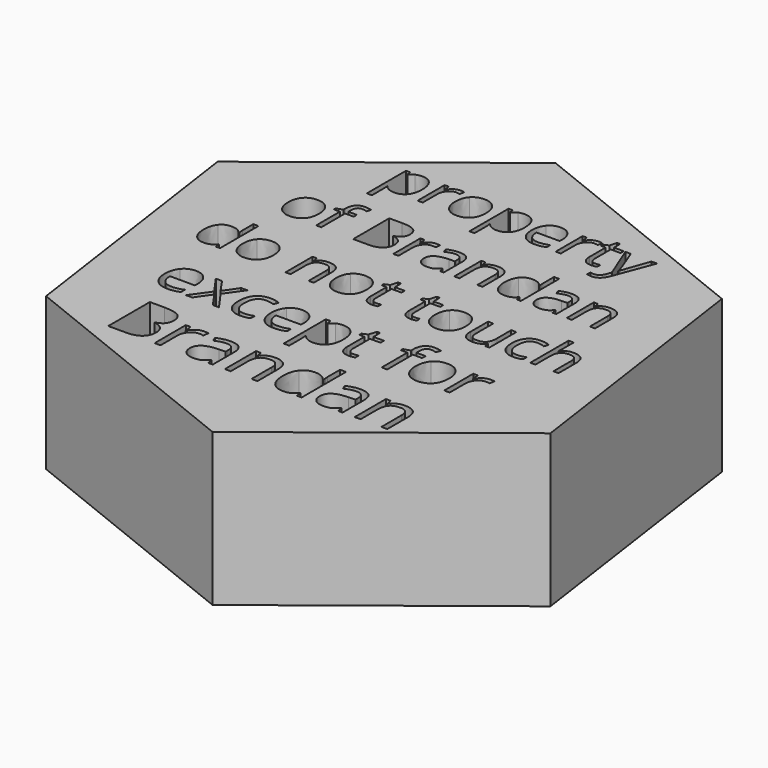
from build123d import *

# Parameters (mm, degrees)
F1_DEPTH = 25.4


with BuildPart() as f1:
    # F0 (on Top) → F1 (new body)
    with BuildSketch(Plane.XY):
        Polygon((34.5890131709, 27.1860289095), (-6.2492850782, 43.5479785525), (-40.838298249, 16.3619496431), (-34.5890131709, -27.1860289095), (6.2492850782, -43.5479785525), (40.838298249, -16.3619496431), align=None)
        with BuildLine():
            Line((-23.000744954, -28.7103280425), (-23.000744954, -20.0400733108))
            Line((-23.000744954, -20.0400733108), (-20.5509093535, -20.0400733108))
            add(Edge.make_bspline(
                [(-20.5509093535, -20.0400733108), (-18.8259670136, -20.0400733108), (-18.0545819078, -20.5562276743)],
                knots=[0, 0, 0, 1, 1, 1], degree=2))
            add(Edge.make_bspline(
                [(-18.0545819078, -20.5562276743), (-17.283196802, -21.0723820379), (-17.283196802, -22.1862886974)],
                knots=[0, 0, 0, 1, 1, 1], degree=2))
            add(Edge.make_bspline(
                [(-17.283196802, -22.1862886974), (-17.283196802, -22.9586226164), (-17.7130091672, -23.4595959692)],
                knots=[0, 0, 0, 1, 1, 1], degree=2))
            add(Edge.make_bspline(
                [(-17.7130091672, -23.4595959692), (-18.1428215324, -23.9605693221), (-18.9682889888, -24.1085841763)],
                knots=[0, 0, 0, 1, 1, 1], degree=2))
            Line((-18.9682889888, -24.1085841763), (-18.9682889888, -24.1674105928))
            add(Edge.make_bspline(
                [(-18.9682889888, -24.1674105928), (-16.9928599725, -24.5051880807), (-16.9928599725, -26.243413805)],
                knots=[0, 0, 0, 1, 1, 1], degree=2))
            add(Edge.make_bspline(
                [(-16.9928599725, -26.243413805), (-16.9928599725, -27.404761123), (-17.7784772758, -28.0575445827)],
                knots=[0, 0, 0, 1, 1, 1], degree=2))
            add(Edge.make_bspline(
                [(-17.7784772758, -28.0575445827), (-18.5640945791, -28.7103280425), (-19.9759285735, -28.7103280425)],
                knots=[0, 0, 0, 1, 1, 1], degree=2))
            Line((-19.9759285735, -28.7103280425), (-23.000744954, -28.7103280425))
        make_face(mode=Mode.SUBTRACT)
        with BuildLine():
            add(Edge.make_bspline(
                [(-13.4348105914, -22.4358265607), (-12.9243491069, -22.0914073806), (-12.3133134265, -22.0914073806)],
                knots=[0, 0, 0, 1, 1, 1], degree=2))
            add(Edge.make_bspline(
                [(-12.3133134265, -22.0914073806), (-11.8806546218, -22.0914073806), (-11.5371842548, -22.1635171814)],
                knots=[0, 0, 0, 1, 1, 1], degree=2))
            Line((-11.5371842548, -22.1635171814), (-11.6738133511, -23.0762754493))
            add(Edge.make_bspline(
                [(-11.6738133511, -23.0762754493), (-12.0761101344, -22.9870870114), (-12.3854232273, -22.9870870114)],
                knots=[0, 0, 0, 1, 1, 1], degree=2))
            add(Edge.make_bspline(
                [(-12.3854232273, -22.9870870114), (-13.1748357833, -22.9870870114), (-13.7346355526, -23.6275359)],
                knots=[0, 0, 0, 1, 1, 1], degree=2))
            add(Edge.make_bspline(
                [(-13.7346355526, -23.6275359), (-14.2944353219, -24.2679847886), (-14.2944353219, -25.2224908359)],
                knots=[0, 0, 0, 1, 1, 1], degree=2))
            Line((-14.2944353219, -25.2224908359), (-14.2944353219, -28.7103280425))
            Line((-14.2944353219, -28.7103280425), (-15.2793033905, -28.7103280425))
            Line((-15.2793033905, -28.7103280425), (-15.2793033905, -22.2109578398))
            Line((-15.2793033905, -22.2109578398), (-14.4671193185, -22.2109578398))
            Line((-14.4671193185, -22.2109578398), (-14.3532617383, -23.4140529372))
            Line((-14.3532617383, -23.4140529372), (-14.3058210799, -23.4140529372))
            add(Edge.make_bspline(
                [(-14.3058210799, -23.4140529372), (-13.9452720759, -22.7802457408), (-13.4348105914, -22.4358265607)],
                knots=[0, 0, 0, 1, 1, 1], degree=2))
        make_face(mode=Mode.SUBTRACT)
        with BuildLine():
            Line((-5.5938185687, -28.7103280425), (-6.3244047083, -28.7103280425))
            Line((-6.3244047083, -28.7103280425), (-6.519860221, -27.7842863903))
            Line((-6.519860221, -27.7842863903), (-6.5673008794, -27.7842863903))
            add(Edge.make_bspline(
                [(-6.5673008794, -27.7842863903), (-7.0530932216, -28.3953220706), (-7.5360391242, -28.6126002862)],
                knots=[0, 0, 0, 1, 1, 1], degree=2))
            add(Edge.make_bspline(
                [(-7.5360391242, -28.6126002862), (-8.0189850269, -28.8298785017), (-8.7438782874, -28.8298785017)],
                knots=[0, 0, 0, 1, 1, 1], degree=2))
            add(Edge.make_bspline(
                [(-8.7438782874, -28.8298785017), (-9.7097700927, -28.8298785017), (-10.258184104, -28.3308027752)],
                knots=[0, 0, 0, 1, 1, 1], degree=2))
            add(Edge.make_bspline(
                [(-10.258184104, -28.3308027752), (-10.8065981153, -27.8317270487), (-10.8065981153, -26.9132759018)],
                knots=[0, 0, 0, 1, 1, 1], degree=2))
            add(Edge.make_bspline(
                [(-10.8065981153, -26.9132759018), (-10.8065981153, -24.9454373908), (-7.6584360229, -24.8505560739)],
                knots=[0, 0, 0, 1, 1, 1], degree=2))
            Line((-7.6584360229, -24.8505560739), (-6.5559151214, -24.8145011735))
            Line((-6.5559151214, -24.8145011735), (-6.5559151214, -24.4103067639))
            add(Edge.make_bspline(
                [(-6.5559151214, -24.4103067639), (-6.5559151214, -23.6455633502), (-6.8842044776, -23.2812190936)],
                knots=[0, 0, 0, 1, 1, 1], degree=2))
            add(Edge.make_bspline(
                [(-6.8842044776, -23.2812190936), (-7.2124938338, -22.916874837), (-7.9373870944, -22.916874837)],
                knots=[0, 0, 0, 1, 1, 1], degree=2))
            add(Edge.make_bspline(
                [(-7.9373870944, -22.916874837), (-8.7495711664, -22.916874837), (-9.7742893882, -23.4140529372)],
                knots=[0, 0, 0, 1, 1, 1], degree=2))
            Line((-9.7742893882, -23.4140529372), (-10.077909602, -22.6606952816))
            add(Edge.make_bspline(
                [(-10.077909602, -22.6606952816), (-9.5978101389, -22.4007204734), (-9.0256757984, -22.2527056192)],
                knots=[0, 0, 0, 1, 1, 1], degree=2))
            add(Edge.make_bspline(
                [(-9.0256757984, -22.2527056192), (-8.4535414579, -22.1046907649), (-7.8766630516, -22.1046907649)],
                knots=[0, 0, 0, 1, 1, 1], degree=2))
            add(Edge.make_bspline(
                [(-7.8766630516, -22.1046907649), (-6.7153157336, -22.1046907649), (-6.1545671512, -22.6198963153)],
                knots=[0, 0, 0, 1, 1, 1], degree=2))
            add(Edge.make_bspline(
                [(-6.1545671512, -22.6198963153), (-5.5938185687, -23.1351018657), (-5.5938185687, -24.2736776676)],
                knots=[0, 0, 0, 1, 1, 1], degree=2))
            Line((-5.5938185687, -24.2736776676), (-5.5938185687, -28.7103280425))
        make_face(mode=Mode.SUBTRACT)
        with BuildLine():
            Line((1.8657505603, -28.7103280425), (0.8808824916, -28.7103280425))
            Line((0.8808824916, -28.7103280425), (0.8808824916, -24.5051880807))
            add(Edge.make_bspline(
                [(0.8808824916, -24.5051880807), (0.8808824916, -23.711980272), (0.5193846745, -23.3201204335)],
                knots=[0, 0, 0, 1, 1, 1], degree=2))
            add(Edge.make_bspline(
                [(0.5193846745, -23.3201204335), (0.1578868574, -22.928260595), (-0.6144470616, -22.928260595)],
                knots=[0, 0, 0, 1, 1, 1], degree=2))
            add(Edge.make_bspline(
                [(-0.6144470616, -22.928260595), (-1.6334724043, -22.928260595), (-2.1078789885, -23.4795210458)],
                knots=[0, 0, 0, 1, 1, 1], degree=2))
            add(Edge.make_bspline(
                [(-2.1078789885, -23.4795210458), (-2.5822855726, -24.0307814965), (-2.5822855726, -25.3002935157)],
                knots=[0, 0, 0, 1, 1, 1], degree=2))
            Line((-2.5822855726, -25.3002935157), (-2.5822855726, -28.7103280425))
            Line((-2.5822855726, -28.7103280425), (-3.5671536413, -28.7103280425))
            Line((-3.5671536413, -28.7103280425), (-3.5671536413, -22.2109578398))
            Line((-3.5671536413, -22.2109578398), (-2.7663553273, -22.2109578398))
            Line((-2.7663553273, -22.2109578398), (-2.606954715, -23.1009445916))
            Line((-2.606954715, -23.1009445916), (-2.5595140566, -23.1009445916))
            add(Edge.make_bspline(
                [(-2.5595140566, -23.1009445916), (-2.2558938427, -22.6208451285), (-1.710326271, -22.3561262545)],
                knots=[0, 0, 0, 1, 1, 1], degree=2))
            add(Edge.make_bspline(
                [(-1.710326271, -22.3561262545), (-1.1647586992, -22.0914073806), (-0.4948966024, -22.0914073806)],
                knots=[0, 0, 0, 1, 1, 1], degree=2))
            add(Edge.make_bspline(
                [(-0.4948966024, -22.0914073806), (0.6797340999, -22.0914073806), (1.2727423301, -22.657848842)],
                knots=[0, 0, 0, 1, 1, 1], degree=2))
            add(Edge.make_bspline(
                [(1.2727423301, -22.657848842), (1.8657505603, -23.2242903035), (1.8657505603, -24.4710308066)],
                knots=[0, 0, 0, 1, 1, 1], degree=2))
            Line((1.8657505603, -24.4710308066), (1.8657505603, -28.7103280425))
        make_face(mode=Mode.SUBTRACT)
        with BuildLine():
            add(Edge.make_bspline(
                [(-22.5217888801, -15.6134171072), (-22.9557129011, -15.7055152667), (-23.5702910043, -15.7055152667)],
                knots=[0, 0, 0, 1, 1, 1], degree=2))
            add(Edge.make_bspline(
                [(-23.5702910043, -15.7055152667), (-24.9145699102, -15.7055152667), (-25.6929764704, -14.885487423)],
                knots=[0, 0, 0, 1, 1, 1], degree=2))
            add(Edge.make_bspline(
                [(-25.6929764704, -14.885487423), (-26.4713830305, -14.0654595792), (-26.4713830305, -12.6113713292)],
                knots=[0, 0, 0, 1, 1, 1], degree=2))
            add(Edge.make_bspline(
                [(-26.4713830305, -12.6113713292), (-26.4713830305, -11.1431141316), (-25.7487667016, -10.2796938857)],
                knots=[0, 0, 0, 1, 1, 1], degree=2))
            add(Edge.make_bspline(
                [(-25.7487667016, -10.2796938857), (-25.0261503728, -9.4162736398), (-23.8076208771, -9.4162736398)],
                knots=[0, 0, 0, 1, 1, 1], degree=2))
            add(Edge.make_bspline(
                [(-23.8076208771, -9.4162736398), (-22.6687917117, -9.4162736398), (-22.0046222918, -10.1663423047)],
                knots=[0, 0, 0, 1, 1, 1], degree=2))
            add(Edge.make_bspline(
                [(-22.0046222918, -10.1663423047), (-21.3404528719, -10.9164109696), (-21.3404528719, -12.145567176)],
                knots=[0, 0, 0, 1, 1, 1], degree=2))
            Line((-21.3404528719, -12.145567176), (-21.3404528719, -12.7264940287))
            Line((-21.3404528719, -12.7264940287), (-25.5185213027, -12.7264940287))
            add(Edge.make_bspline(
                [(-25.5185213027, -12.7264940287), (-25.4901834075, -13.7944784559), (-24.9783301745, -14.3479529725)],
                knots=[0, 0, 0, 1, 1, 1], degree=2))
            add(Edge.make_bspline(
                [(-24.9783301745, -14.3479529725), (-24.4664769416, -14.901427489), (-23.5366397537, -14.901427489)],
                knots=[0, 0, 0, 1, 1, 1], degree=2))
            add(Edge.make_bspline(
                [(-23.5366397537, -14.901427489), (-22.5572112492, -14.901427489), (-21.6008072845, -14.4922991264)],
                knots=[0, 0, 0, 1, 1, 1], degree=2))
            Line((-21.6008072845, -14.4922991264), (-21.6008072845, -15.3123269702))
            add(Edge.make_bspline(
                [(-21.6008072845, -15.3123269702), (-22.0878648591, -15.5213189476), (-22.5217888801, -15.6134171072)],
                knots=[0, 0, 0, 1, 1, 1], degree=2))
        make_face(mode=Mode.SUBTRACT)
        Polygon((-20.5310517388, -15.5939348042), (-18.3118403171, -12.4891641559), (-20.4212423948, -9.5278541024), (-19.374511389, -9.5278541024), (-17.7751914259, -11.8515615128), (-16.1811848181, -9.5278541024), (-15.145080523, -9.5278541024), (-17.2544826006, -12.4891641559), (-15.0352711789, -15.5939348042), (-16.0749177109, -15.5939348042), (-17.7751914259, -13.1356223913), (-19.4914052069, -15.5939348042), align=None, mode=Mode.SUBTRACT)
        with BuildLine():
            add(Edge.make_bspline(
                [(-9.8777742436, -15.3884850636), (-10.485267873, -15.7055152667), (-11.4097917055, -15.7055152667)],
                knots=[0, 0, 0, 1, 1, 1], degree=2))
            add(Edge.make_bspline(
                [(-11.4097917055, -15.7055152667), (-12.7275038346, -15.7055152667), (-13.4501201634, -14.8943430152)],
                knots=[0, 0, 0, 1, 1, 1], degree=2))
            add(Edge.make_bspline(
                [(-13.4501201634, -14.8943430152), (-14.1727364923, -14.0831707637), (-14.1727364923, -12.5989735)],
                knots=[0, 0, 0, 1, 1, 1], degree=2))
            add(Edge.make_bspline(
                [(-14.1727364923, -12.5989735), (-14.1727364923, -11.0775827488), (-13.4386078935, -10.2469281943)],
                knots=[0, 0, 0, 1, 1, 1], degree=2))
            add(Edge.make_bspline(
                [(-13.4386078935, -10.2469281943), (-12.7044792947, -9.4162736398), (-11.3495736781, -9.4162736398)],
                knots=[0, 0, 0, 1, 1, 1], degree=2))
            add(Edge.make_bspline(
                [(-11.3495736781, -9.4162736398), (-10.9121074202, -9.4162736398), (-10.4746411622, -9.5110284771)],
                knots=[0, 0, 0, 1, 1, 1], degree=2))
            add(Edge.make_bspline(
                [(-10.4746411622, -9.5110284771), (-10.0371749043, -9.6057833143), (-9.7892183209, -9.7333038429)],
                knots=[0, 0, 0, 1, 1, 1], degree=2))
            Line((-9.7892183209, -9.7333038429), (-10.0708261549, -10.5125959623))
            add(Edge.make_bspline(
                [(-10.0708261549, -10.5125959623), (-10.3754585289, -10.390388789), (-10.7349955748, -10.3106884587)],
                knots=[0, 0, 0, 1, 1, 1], degree=2))
            add(Edge.make_bspline(
                [(-10.7349955748, -10.3106884587), (-11.0945326208, -10.2309881283), (-11.3708270995, -10.2309881283)],
                knots=[0, 0, 0, 1, 1, 1], degree=2))
            add(Edge.make_bspline(
                [(-11.3708270995, -10.2309881283), (-13.2198747645, -10.2309881283), (-13.2198747645, -12.5883467893)],
                knots=[0, 0, 0, 1, 1, 1], degree=2))
            add(Edge.make_bspline(
                [(-13.2198747645, -12.5883467893), (-13.2198747645, -13.7059225332), (-12.7691251182, -14.3036750111)],
                knots=[0, 0, 0, 1, 1, 1], degree=2))
            add(Edge.make_bspline(
                [(-12.7691251182, -14.3036750111), (-12.3183754719, -14.901427489), (-11.4328162454, -14.901427489)],
                knots=[0, 0, 0, 1, 1, 1], degree=2))
            add(Edge.make_bspline(
                [(-11.4328162454, -14.901427489), (-10.6747775474, -14.901427489), (-9.8777742436, -14.5755416937)],
                knots=[0, 0, 0, 1, 1, 1], degree=2))
            Line((-9.8777742436, -14.5755416937), (-9.8777742436, -15.3884850636))
        make_face(mode=Mode.SUBTRACT)
        with BuildLine():
            add(Edge.make_bspline(
                [(-4.8265444154, -15.6134171072), (-5.2604684364, -15.7055152667), (-5.8750465396, -15.7055152667)],
                knots=[0, 0, 0, 1, 1, 1], degree=2))
            add(Edge.make_bspline(
                [(-5.8750465396, -15.7055152667), (-7.2193254455, -15.7055152667), (-7.9977320056, -14.885487423)],
                knots=[0, 0, 0, 1, 1, 1], degree=2))
            add(Edge.make_bspline(
                [(-7.9977320056, -14.885487423), (-8.7761385657, -14.0654595792), (-8.7761385657, -12.6113713292)],
                knots=[0, 0, 0, 1, 1, 1], degree=2))
            add(Edge.make_bspline(
                [(-8.7761385657, -12.6113713292), (-8.7761385657, -11.1431141316), (-8.0535222369, -10.2796938857)],
                knots=[0, 0, 0, 1, 1, 1], degree=2))
            add(Edge.make_bspline(
                [(-8.0535222369, -10.2796938857), (-7.330905908, -9.4162736398), (-6.1123764123, -9.4162736398)],
                knots=[0, 0, 0, 1, 1, 1], degree=2))
            add(Edge.make_bspline(
                [(-6.1123764123, -9.4162736398), (-4.973547247, -9.4162736398), (-4.3093778271, -10.1663423047)],
                knots=[0, 0, 0, 1, 1, 1], degree=2))
            add(Edge.make_bspline(
                [(-4.3093778271, -10.1663423047), (-3.6452084072, -10.9164109696), (-3.6452084072, -12.145567176)],
                knots=[0, 0, 0, 1, 1, 1], degree=2))
            Line((-3.6452084072, -12.145567176), (-3.6452084072, -12.7264940287))
            Line((-3.6452084072, -12.7264940287), (-7.823276838, -12.7264940287))
            add(Edge.make_bspline(
                [(-7.823276838, -12.7264940287), (-7.7949389427, -13.7944784559), (-7.2830857098, -14.3479529725)],
                knots=[0, 0, 0, 1, 1, 1], degree=2))
            add(Edge.make_bspline(
                [(-7.2830857098, -14.3479529725), (-6.7712324768, -14.901427489), (-5.841395289, -14.901427489)],
                knots=[0, 0, 0, 1, 1, 1], degree=2))
            add(Edge.make_bspline(
                [(-5.841395289, -14.901427489), (-4.8619667844, -14.901427489), (-3.9055628198, -14.4922991264)],
                knots=[0, 0, 0, 1, 1, 1], degree=2))
            Line((-3.9055628198, -14.4922991264), (-3.9055628198, -15.3123269702))
            add(Edge.make_bspline(
                [(-3.9055628198, -15.3123269702), (-4.3926203944, -15.5213189476), (-4.8265444154, -15.6134171072)],
                knots=[0, 0, 0, 1, 1, 1], degree=2))
        make_face(mode=Mode.SUBTRACT)
        with BuildLine():
            Line((8.4410258165, -28.7103280425), (8.3100895992, -27.839317554))
            Line((8.3100895992, -27.839317554), (8.2569560618, -27.839317554))
            add(Edge.make_bspline(
                [(8.2569560618, -27.839317554), (7.575708207, -28.8298785017), (6.21700775, -28.8298785017)],
                knots=[0, 0, 0, 1, 1, 1], degree=2))
            add(Edge.make_bspline(
                [(6.21700775, -28.8298785017), (4.9418028518, -28.8298785017), (4.2330394151, -27.9579192001)],
                knots=[0, 0, 0, 1, 1, 1], degree=2))
            add(Edge.make_bspline(
                [(4.2330394151, -27.9579192001), (3.5242759784, -27.0859598984), (3.5242759784, -25.4786703913)],
                knots=[0, 0, 0, 1, 1, 1], degree=2))
            add(Edge.make_bspline(
                [(3.5242759784, -25.4786703913), (3.5242759784, -23.8713808843), (4.2358858546, -22.9813941324)],
                knots=[0, 0, 0, 1, 1, 1], degree=2))
            add(Edge.make_bspline(
                [(4.2358858546, -22.9813941324), (4.9474957309, -22.0914073806), (6.21700775, -22.0914073806)],
                knots=[0, 0, 0, 1, 1, 1], degree=2))
            add(Edge.make_bspline(
                [(6.21700775, -22.0914073806), (7.5396533066, -22.0914073806), (8.2455703038, -23.0535039332)],
                knots=[0, 0, 0, 1, 1, 1], degree=2))
            Line((8.2455703038, -23.0535039332), (8.3233729836, -23.0535039332))
            Line((8.3233729836, -23.0535039332), (8.2816252042, -22.5847902281))
            Line((8.2816252042, -22.5847902281), (8.2569560618, -22.127462281))
            Line((8.2569560618, -22.127462281), (8.2569560618, -19.4821711678))
            Line((8.2569560618, -19.4821711678), (9.2418241305, -19.4821711678))
            Line((9.2418241305, -19.4821711678), (9.2418241305, -28.7103280425))
            Line((9.2418241305, -28.7103280425), (8.4410258165, -28.7103280425))
        make_face(mode=Mode.SUBTRACT)
        with BuildLine():
            Line((16.0562003051, -28.7103280425), (15.3256141655, -28.7103280425))
            Line((15.3256141655, -28.7103280425), (15.1301586528, -27.7842863903))
            Line((15.1301586528, -27.7842863903), (15.0827179944, -27.7842863903))
            add(Edge.make_bspline(
                [(15.0827179944, -27.7842863903), (14.5969256523, -28.3953220706), (14.1139797496, -28.6126002862)],
                knots=[0, 0, 0, 1, 1, 1], degree=2))
            add(Edge.make_bspline(
                [(14.1139797496, -28.6126002862), (13.631033847, -28.8298785017), (12.9061405864, -28.8298785017)],
                knots=[0, 0, 0, 1, 1, 1], degree=2))
            add(Edge.make_bspline(
                [(12.9061405864, -28.8298785017), (11.9402487811, -28.8298785017), (11.3918347698, -28.3308027752)],
                knots=[0, 0, 0, 1, 1, 1], degree=2))
            add(Edge.make_bspline(
                [(11.3918347698, -28.3308027752), (10.8434207585, -27.8317270487), (10.8434207585, -26.9132759018)],
                knots=[0, 0, 0, 1, 1, 1], degree=2))
            add(Edge.make_bspline(
                [(10.8434207585, -26.9132759018), (10.8434207585, -24.9454373908), (13.9915828509, -24.8505560739)],
                knots=[0, 0, 0, 1, 1, 1], degree=2))
            Line((13.9915828509, -24.8505560739), (15.0941037524, -24.8145011735))
            Line((15.0941037524, -24.8145011735), (15.0941037524, -24.4103067639))
            add(Edge.make_bspline(
                [(15.0941037524, -24.4103067639), (15.0941037524, -23.6455633502), (14.7658143962, -23.2812190936)],
                knots=[0, 0, 0, 1, 1, 1], degree=2))
            add(Edge.make_bspline(
                [(14.7658143962, -23.2812190936), (14.43752504, -22.916874837), (13.7126317794, -22.916874837)],
                knots=[0, 0, 0, 1, 1, 1], degree=2))
            add(Edge.make_bspline(
                [(13.7126317794, -22.916874837), (12.9004477074, -22.916874837), (11.8757294856, -23.4140529372)],
                knots=[0, 0, 0, 1, 1, 1], degree=2))
            Line((11.8757294856, -23.4140529372), (11.5721092718, -22.6606952816))
            add(Edge.make_bspline(
                [(11.5721092718, -22.6606952816), (12.0522087349, -22.4007204734), (12.6243430754, -22.2527056192)],
                knots=[0, 0, 0, 1, 1, 1], degree=2))
            add(Edge.make_bspline(
                [(12.6243430754, -22.2527056192), (13.1964774159, -22.1046907649), (13.7733558222, -22.1046907649)],
                knots=[0, 0, 0, 1, 1, 1], degree=2))
            add(Edge.make_bspline(
                [(13.7733558222, -22.1046907649), (14.9347031402, -22.1046907649), (15.4954517226, -22.6198963153)],
                knots=[0, 0, 0, 1, 1, 1], degree=2))
            add(Edge.make_bspline(
                [(15.4954517226, -22.6198963153), (16.0562003051, -23.1351018657), (16.0562003051, -24.2736776676)],
                knots=[0, 0, 0, 1, 1, 1], degree=2))
            Line((16.0562003051, -24.2736776676), (16.0562003051, -28.7103280425))
        make_face(mode=Mode.SUBTRACT)
        with BuildLine():
            Line((23.5157694341, -28.7103280425), (22.5309013654, -28.7103280425))
            Line((22.5309013654, -28.7103280425), (22.5309013654, -24.5051880807))
            add(Edge.make_bspline(
                [(22.5309013654, -24.5051880807), (22.5309013654, -23.711980272), (22.1694035483, -23.3201204335)],
                knots=[0, 0, 0, 1, 1, 1], degree=2))
            add(Edge.make_bspline(
                [(22.1694035483, -23.3201204335), (21.8079057312, -22.928260595), (21.0355718122, -22.928260595)],
                knots=[0, 0, 0, 1, 1, 1], degree=2))
            add(Edge.make_bspline(
                [(21.0355718122, -22.928260595), (20.0165464695, -22.928260595), (19.5421398853, -23.4795210458)],
                knots=[0, 0, 0, 1, 1, 1], degree=2))
            add(Edge.make_bspline(
                [(19.5421398853, -23.4795210458), (19.0677333012, -24.0307814965), (19.0677333012, -25.3002935157)],
                knots=[0, 0, 0, 1, 1, 1], degree=2))
            Line((19.0677333012, -25.3002935157), (19.0677333012, -28.7103280425))
            Line((19.0677333012, -28.7103280425), (18.0828652325, -28.7103280425))
            Line((18.0828652325, -28.7103280425), (18.0828652325, -22.2109578398))
            Line((18.0828652325, -22.2109578398), (18.8836635466, -22.2109578398))
            Line((18.8836635466, -22.2109578398), (19.0430641588, -23.1009445916))
            Line((19.0430641588, -23.1009445916), (19.0905048172, -23.1009445916))
            add(Edge.make_bspline(
                [(19.0905048172, -23.1009445916), (19.3941250311, -22.6208451285), (19.9396926028, -22.3561262545)],
                knots=[0, 0, 0, 1, 1, 1], degree=2))
            add(Edge.make_bspline(
                [(19.9396926028, -22.3561262545), (20.4852601746, -22.0914073806), (21.1551222714, -22.0914073806)],
                knots=[0, 0, 0, 1, 1, 1], degree=2))
            add(Edge.make_bspline(
                [(21.1551222714, -22.0914073806), (22.3297529737, -22.0914073806), (22.9227612039, -22.657848842)],
                knots=[0, 0, 0, 1, 1, 1], degree=2))
            add(Edge.make_bspline(
                [(22.9227612039, -22.657848842), (23.5157694341, -23.2242903035), (23.5157694341, -24.4710308066)],
                knots=[0, 0, 0, 1, 1, 1], degree=2))
            Line((23.5157694341, -24.4710308066), (23.5157694341, -28.7103280425))
        make_face(mode=Mode.SUBTRACT)
        with BuildLine():
            add(Edge.make_bspline(
                [(2.5970985807, -14.8775173899), (1.9302724832, -15.7055152667), (0.745394238, -15.7055152667)],
                knots=[0, 0, 0, 1, 1, 1], degree=2))
            add(Edge.make_bspline(
                [(0.745394238, -15.7055152667), (0.1520695563, -15.7055152667), (-0.337644696, -15.4867821378)],
                knots=[0, 0, 0, 1, 1, 1], degree=2))
            add(Edge.make_bspline(
                [(-0.337644696, -15.4867821378), (-0.8273589483, -15.2680490088), (-1.158558099, -14.8128715664)],
                knots=[0, 0, 0, 1, 1, 1], degree=2))
            Line((-1.158558099, -14.8128715664), (-1.2258606002, -14.8128715664))
            add(Edge.make_bspline(
                [(-1.2258606002, -14.8128715664), (-1.158558099, -15.3442071023), (-1.158558099, -15.8206379662)],
                knots=[0, 0, 0, 1, 1, 1], degree=2))
            Line((-1.158558099, -15.8206379662), (-1.158558099, -18.317914985))
            Line((-1.158558099, -18.317914985), (-2.0777685762, -18.317914985))
            Line((-2.0777685762, -18.317914985), (-2.0777685762, -9.5278541024))
            Line((-2.0777685762, -9.5278541024), (-1.330356589, -9.5278541024))
            Line((-1.330356589, -9.5278541024), (-1.2028360604, -10.3585086569))
            Line((-1.2028360604, -10.3585086569), (-1.158558099, -10.3585086569))
            add(Edge.make_bspline(
                [(-1.158558099, -10.3585086569), (-0.8043344084, -9.8590532531), (-0.3341024591, -9.6376634465)],
                knots=[0, 0, 0, 1, 1, 1], degree=2))
            add(Edge.make_bspline(
                [(-0.3341024591, -9.6376634465), (0.1361294902, -9.4162736398), (0.745394238, -9.4162736398)],
                knots=[0, 0, 0, 1, 1, 1], degree=2))
            add(Edge.make_bspline(
                [(0.745394238, -9.4162736398), (1.9515259046, -9.4162736398), (2.6077252915, -10.241614839)],
                knots=[0, 0, 0, 1, 1, 1], degree=2))
            add(Edge.make_bspline(
                [(2.6077252915, -10.241614839), (3.2639246783, -11.0669560381), (3.2639246783, -12.5546955387)],
                knots=[0, 0, 0, 1, 1, 1], degree=2))
            add(Edge.make_bspline(
                [(3.2639246783, -12.5546955387), (3.2639246783, -14.0495195131), (2.5970985807, -14.8775173899)],
                knots=[0, 0, 0, 1, 1, 1], degree=2))
        make_face(mode=Mode.SUBTRACT)
        with BuildLine():
            add(Edge.make_bspline(
                [(6.1136542693, -14.6525853464), (6.3740086819, -14.9457054504), (6.8274150059, -14.9457054504)],
                knots=[0, 0, 0, 1, 1, 1], degree=2))
            add(Edge.make_bspline(
                [(6.8274150059, -14.9457054504), (7.0718293525, -14.9457054504), (7.2985325144, -14.9102830813)],
                knots=[0, 0, 0, 1, 1, 1], degree=2))
            add(Edge.make_bspline(
                [(7.2985325144, -14.9102830813), (7.5252356764, -14.8748607122), (7.6580695604, -14.8358961063)],
                knots=[0, 0, 0, 1, 1, 1], degree=2))
            Line((7.6580695604, -14.8358961063), (7.6580695604, -15.5390301322))
            add(Edge.make_bspline(
                [(7.6580695604, -15.5390301322), (7.5092956104, -15.6098748703), (7.2188321841, -15.6576950685)],
                knots=[0, 0, 0, 1, 1, 1], degree=2))
            add(Edge.make_bspline(
                [(7.2188321841, -15.6576950685), (6.9283687578, -15.7055152667), (6.6945811219, -15.7055152667)],
                knots=[0, 0, 0, 1, 1, 1], degree=2))
            add(Edge.make_bspline(
                [(6.6945811219, -15.7055152667), (4.935860498, -15.7055152667), (4.935860498, -13.8511542464)],
                knots=[0, 0, 0, 1, 1, 1], degree=2))
            Line((4.935860498, -13.8511542464), (4.935860498, -10.241614839))
            Line((4.935860498, -10.241614839), (4.0662413376, -10.241614839))
            Line((4.0662413376, -10.241614839), (4.0662413376, -9.7988352257))
            Line((4.0662413376, -9.7988352257), (4.935860498, -9.4162736398))
            Line((4.935860498, -9.4162736398), (5.3219643208, -8.1215860506))
            Line((5.3219643208, -8.1215860506), (5.8532998567, -8.1215860506))
            Line((5.8532998567, -8.1215860506), (5.8532998567, -9.5278541024))
            Line((5.8532998567, -9.5278541024), (7.6137915991, -9.5278541024))
            Line((7.6137915991, -9.5278541024), (7.6137915991, -10.241614839))
            Line((7.6137915991, -10.241614839), (5.8532998567, -10.241614839))
            Line((5.8532998567, -10.241614839), (5.8532998567, -13.8121896404))
            add(Edge.make_bspline(
                [(5.8532998567, -13.8121896404), (5.8532998567, -14.3594652424), (6.1136542693, -14.6525853464)],
                knots=[0, 0, 0, 1, 1, 1], degree=2))
        make_face(mode=Mode.SUBTRACT)
        with BuildLine():
            Line((14.5494914614, -9.5278541024), (14.5494914614, -10.241614839))
            Line((14.5494914614, -10.241614839), (13.0050761703, -10.241614839))
            Line((13.0050761703, -10.241614839), (13.0050761703, -15.5939348042))
            Line((13.0050761703, -15.5939348042), (12.0858656931, -15.5939348042))
            Line((12.0858656931, -15.5939348042), (12.0858656931, -10.241614839))
            Line((12.0858656931, -10.241614839), (11.0019411998, -10.241614839))
            Line((11.0019411998, -10.241614839), (11.0019411998, -9.827173121))
            Line((11.0019411998, -9.827173121), (12.0858656931, -9.4942028518))
            Line((12.0858656931, -9.4942028518), (12.0858656931, -9.1576903457))
            add(Edge.make_bspline(
                [(12.0858656931, -9.1576903457), (12.0858656931, -6.9207677395), (14.0394093469, -6.9207677395)],
                knots=[0, 0, 0, 1, 1, 1], degree=2))
            add(Edge.make_bspline(
                [(14.0394093469, -6.9207677395), (14.5211535661, -6.9207677395), (15.1693829199, -7.1138196508)],
                knots=[0, 0, 0, 1, 1, 1], degree=2))
            Line((15.1693829199, -7.1138196508), (14.9302819288, -7.8506049273))
            add(Edge.make_bspline(
                [(14.9302819288, -7.8506049273), (14.3989463929, -7.6788064374), (14.0234692808, -7.6788064374)],
                knots=[0, 0, 0, 1, 1, 1], degree=2))
            add(Edge.make_bspline(
                [(14.0234692808, -7.6788064374), (13.5027604556, -7.6788064374), (13.2539183129, -8.025060095)],
                knots=[0, 0, 0, 1, 1, 1], degree=2))
            add(Edge.make_bspline(
                [(13.2539183129, -8.025060095), (13.0050761703, -8.3713137525), (13.0050761703, -9.1346658058)],
                knots=[0, 0, 0, 1, 1, 1], degree=2))
            Line((13.0050761703, -9.1346658058), (13.0050761703, -9.5278541024))
            Line((13.0050761703, -9.5278541024), (14.5494914614, -9.5278541024))
        make_face(mode=Mode.SUBTRACT)
        with BuildLine():
            add(Edge.make_bspline(
                [(20.141797977, -10.2637538196), (20.8918666419, -11.1112339994), (20.8918666419, -12.5546955387)],
                knots=[0, 0, 0, 1, 1, 1], degree=2))
            add(Edge.make_bspline(
                [(20.8918666419, -12.5546955387), (20.8918666419, -14.0388928024), (20.1453402139, -14.8722040346)],
                knots=[0, 0, 0, 1, 1, 1], degree=2))
            add(Edge.make_bspline(
                [(20.1453402139, -14.8722040346), (19.3988137859, -15.7055152667), (18.0811016568, -15.7055152667)],
                knots=[0, 0, 0, 1, 1, 1], degree=2))
            add(Edge.make_bspline(
                [(18.0811016568, -15.7055152667), (17.2663871684, -15.7055152667), (16.6358689991, -15.3229536809)],
                knots=[0, 0, 0, 1, 1, 1], degree=2))
            add(Edge.make_bspline(
                [(16.6358689991, -15.3229536809), (16.0053508298, -14.940392095), (15.6617538499, -14.2266313584)],
                knots=[0, 0, 0, 1, 1, 1], degree=2))
            add(Edge.make_bspline(
                [(15.6617538499, -14.2266313584), (15.31815687, -13.5128706218), (15.31815687, -12.5546955387)],
                knots=[0, 0, 0, 1, 1, 1], degree=2))
            add(Edge.make_bspline(
                [(15.31815687, -12.5546955387), (15.31815687, -11.0722693935), (16.0602555018, -10.2442715167)],
                knots=[0, 0, 0, 1, 1, 1], degree=2))
            add(Edge.make_bspline(
                [(16.0602555018, -10.2442715167), (16.8023541337, -9.4162736398), (18.1200662628, -9.4162736398)],
                knots=[0, 0, 0, 1, 1, 1], degree=2))
            add(Edge.make_bspline(
                [(18.1200662628, -9.4162736398), (19.3917293121, -9.4162736398), (20.141797977, -10.2637538196)],
                knots=[0, 0, 0, 1, 1, 1], degree=2))
        make_face(mode=Mode.SUBTRACT)
        with BuildLine():
            add(Edge.make_bspline(
                [(24.2251115706, -9.7377316391), (24.7015424344, -9.4162736398), (25.2718425763, -9.4162736398)],
                knots=[0, 0, 0, 1, 1, 1], degree=2))
            add(Edge.make_bspline(
                [(25.2718425763, -9.4162736398), (25.6756575836, -9.4162736398), (25.9962300236, -9.4835761411)],
                knots=[0, 0, 0, 1, 1, 1], degree=2))
            Line((25.9962300236, -9.4835761411), (25.868709495, -10.335484117))
            add(Edge.make_bspline(
                [(25.868709495, -10.335484117), (25.493232383, -10.2522415497), (25.2045400751, -10.2522415497)],
                knots=[0, 0, 0, 1, 1, 1], degree=2))
            add(Edge.make_bspline(
                [(25.2045400751, -10.2522415497), (24.4677547986, -10.2522415497), (23.945274855, -10.8499940276)],
                knots=[0, 0, 0, 1, 1, 1], degree=2))
            add(Edge.make_bspline(
                [(23.945274855, -10.8499940276), (23.4227949113, -11.4477465055), (23.4227949113, -12.3386190874)],
                knots=[0, 0, 0, 1, 1, 1], degree=2))
            Line((23.4227949113, -12.3386190874), (23.4227949113, -15.5939348042))
            Line((23.4227949113, -15.5939348042), (22.5035844342, -15.5939348042))
            Line((22.5035844342, -15.5939348042), (22.5035844342, -9.5278541024))
            Line((22.5035844342, -9.5278541024), (23.2616231321, -9.5278541024))
            Line((23.2616231321, -9.5278541024), (23.3678902393, -10.6507432016))
            Line((23.3678902393, -10.6507432016), (23.4121682006, -10.6507432016))
            add(Edge.make_bspline(
                [(23.4121682006, -10.6507432016), (23.7486807067, -10.0591896383), (24.2251115706, -9.7377316391)],
                knots=[0, 0, 0, 1, 1, 1], degree=2))
        make_face(mode=Mode.SUBTRACT)
        with BuildLine():
            Line((-26.0447943211, -2.4775429629), (-26.1582723946, -1.7226670825))
            Line((-26.1582723946, -1.7226670825), (-26.204321468, -1.7226670825))
            add(Edge.make_bspline(
                [(-26.204321468, -1.7226670825), (-26.7947363722, -2.5811533778), (-27.9722769612, -2.5811533778)],
                knots=[0, 0, 0, 1, 1, 1], degree=2))
            add(Edge.make_bspline(
                [(-27.9722769612, -2.5811533778), (-29.0774547207, -2.5811533778), (-29.6917164665, -1.8254551926)],
                knots=[0, 0, 0, 1, 1, 1], degree=2))
            add(Edge.make_bspline(
                [(-29.6917164665, -1.8254551926), (-30.3059782123, -1.0697570073), (-30.3059782123, 0.3232274604)],
                knots=[0, 0, 0, 1, 1, 1], degree=2))
            add(Edge.make_bspline(
                [(-30.3059782123, 0.3232274604), (-30.3059782123, 1.7162119281), (-29.6892495519, 2.4875339061)],
                knots=[0, 0, 0, 1, 1, 1], degree=2))
            add(Edge.make_bspline(
                [(-29.6892495519, 2.4875339061), (-29.0725208914, 3.2588558841), (-27.9722769612, 3.2588558841)],
                knots=[0, 0, 0, 1, 1, 1], degree=2))
            add(Edge.make_bspline(
                [(-27.9722769612, 3.2588558841), (-26.8259839577, 3.2588558841), (-26.2141891265, 2.4250387352)],
                knots=[0, 0, 0, 1, 1, 1], degree=2))
            Line((-26.2141891265, 2.4250387352), (-26.1467601263, 2.4250387352))
            Line((-26.1467601263, 2.4250387352), (-26.1829415411, 2.8312573462))
            Line((-26.1829415411, 2.8312573462), (-26.204321468, 3.2276082986))
            Line((-26.204321468, 3.2276082986), (-26.204321468, 5.5201943057))
            Line((-26.204321468, 5.5201943057), (-25.3507690019, 5.5201943057))
            Line((-25.3507690019, 5.5201943057), (-25.3507690019, -2.4775429629))
            Line((-25.3507690019, -2.4775429629), (-26.0447943211, -2.4775429629))
        make_face(mode=Mode.SUBTRACT)
        with BuildLine():
            add(Edge.make_bspline(
                [(-19.3767240445, 2.4719101133), (-18.6802318106, 1.6849643426), (-18.6802318106, 0.3446073873)],
                knots=[0, 0, 0, 1, 1, 1], degree=2))
            add(Edge.make_bspline(
                [(-18.6802318106, 0.3446073873), (-18.6802318106, -1.0335755926), (-19.373434825, -1.8073644852)],
                knots=[0, 0, 0, 1, 1, 1], degree=2))
            add(Edge.make_bspline(
                [(-19.373434825, -1.8073644852), (-20.0666378393, -2.5811533778), (-21.2902275016, -2.5811533778)],
                knots=[0, 0, 0, 1, 1, 1], degree=2))
            add(Edge.make_bspline(
                [(-21.2902275016, -2.5811533778), (-22.0467479917, -2.5811533778), (-22.6322290667, -2.2259176694)],
                knots=[0, 0, 0, 1, 1, 1], degree=2))
            add(Edge.make_bspline(
                [(-22.6322290667, -2.2259176694), (-23.2177101417, -1.870681961), (-23.5367644353, -1.2079042273)],
                knots=[0, 0, 0, 1, 1, 1], degree=2))
            add(Edge.make_bspline(
                [(-23.5367644353, -1.2079042273), (-23.855818729, -0.5451264935), (-23.855818729, 0.3446073873)],
                knots=[0, 0, 0, 1, 1, 1], degree=2))
            add(Edge.make_bspline(
                [(-23.855818729, 0.3446073873), (-23.855818729, 1.7211457574), (-23.1667272391, 2.4900008207)],
                knots=[0, 0, 0, 1, 1, 1], degree=2))
            add(Edge.make_bspline(
                [(-23.1667272391, 2.4900008207), (-22.4776357492, 3.2588558841), (-21.2540460868, 3.2588558841)],
                knots=[0, 0, 0, 1, 1, 1], degree=2))
            add(Edge.make_bspline(
                [(-21.2540460868, 3.2588558841), (-20.0732162783, 3.2588558841), (-19.3767240445, 2.4719101133)],
                knots=[0, 0, 0, 1, 1, 1], degree=2))
        make_face(mode=Mode.SUBTRACT)
        with BuildLine():
            add(Edge.make_bspline(
                [(-22.0377074584, 15.2968281521), (-21.3412155669, 14.5098827682), (-21.3412155669, 13.1695264718)],
                knots=[0, 0, 0, 1, 1, 1], degree=2))
            add(Edge.make_bspline(
                [(-21.3412155669, 13.1695264718), (-21.3412155669, 11.7913441694), (-22.0344182405, 11.0175556571)],
                knots=[0, 0, 0, 1, 1, 1], degree=2))
            add(Edge.make_bspline(
                [(-22.0344182405, 11.0175556571), (-22.727620914, 10.2437671449), (-23.9512099749, 10.2437671449)],
                knots=[0, 0, 0, 1, 1, 1], degree=2))
            add(Edge.make_bspline(
                [(-23.9512099749, 10.2437671449), (-24.7077300931, 10.2437671449), (-25.2932108803, 10.5990026786)],
                knots=[0, 0, 0, 1, 1, 1], degree=2))
            add(Edge.make_bspline(
                [(-25.2932108803, 10.5990026786), (-25.8786916675, 10.9542382124), (-26.1977458043, 11.6170156204)],
                knots=[0, 0, 0, 1, 1, 1], degree=2))
            add(Edge.make_bspline(
                [(-26.1977458043, 11.6170156204), (-26.5167999411, 12.2797930283), (-26.5167999411, 13.1695264718)],
                knots=[0, 0, 0, 1, 1, 1], degree=2))
            add(Edge.make_bspline(
                [(-26.5167999411, 13.1695264718), (-26.5167999411, 14.5460641652), (-25.8277087899, 15.3149188506)],
                knots=[0, 0, 0, 1, 1, 1], degree=2))
            add(Edge.make_bspline(
                [(-25.8277087899, 15.3149188506), (-25.1386176387, 16.083773536), (-23.9150285779, 16.083773536)],
                knots=[0, 0, 0, 1, 1, 1], degree=2))
            add(Edge.make_bspline(
                [(-23.9150285779, 16.083773536), (-22.7341993498, 16.083773536), (-22.0377074584, 15.2968281521)],
                knots=[0, 0, 0, 1, 1, 1], degree=2))
        make_face(mode=Mode.SUBTRACT)
        with BuildLine():
            Line((-9.7401331489, -2.4775429629), (-10.593685615, -2.4775429629))
            Line((-10.593685615, -2.4775429629), (-10.593685615, 1.1669122679))
            add(Edge.make_bspline(
                [(-10.593685615, 1.1669122679), (-10.593685615, 1.854359148), (-10.9069837745, 2.1939710637)],
                knots=[0, 0, 0, 1, 1, 1], degree=2))
            add(Edge.make_bspline(
                [(-10.9069837745, 2.1939710637), (-11.220281934, 2.5335829794), (-11.8896381068, 2.5335829794)],
                knots=[0, 0, 0, 1, 1, 1], degree=2))
            add(Edge.make_bspline(
                [(-11.8896381068, 2.5335829794), (-12.7727935485, 2.5335829794), (-13.1839459888, 2.0558238438)],
                knots=[0, 0, 0, 1, 1, 1], degree=2))
            add(Edge.make_bspline(
                [(-13.1839459888, 2.0558238438), (-13.5950984291, 1.5780647082), (-13.5950984291, 0.4778207779)],
                knots=[0, 0, 0, 1, 1, 1], degree=2))
            Line((-13.5950984291, 0.4778207779), (-13.5950984291, -2.4775429629))
            Line((-13.5950984291, -2.4775429629), (-14.4486508951, -2.4775429629))
            Line((-14.4486508951, -2.4775429629), (-14.4486508951, 3.1552454691))
            Line((-14.4486508951, 3.1552454691), (-13.7546255759, 3.1552454691))
            Line((-13.7546255759, 3.1552454691), (-13.616478356, 2.3839234911))
            Line((-13.616478356, 2.3839234911), (-13.575363112, 2.3839234911))
            add(Edge.make_bspline(
                [(-13.575363112, 2.3839234911), (-13.3122255502, 2.8000097607), (-12.8394002438, 3.0294328224)],
                knots=[0, 0, 0, 1, 1, 1], degree=2))
            add(Edge.make_bspline(
                [(-12.8394002438, 3.0294328224), (-12.3665749375, 3.2588558841), (-11.7860276918, 3.2588558841)],
                knots=[0, 0, 0, 1, 1, 1], degree=2))
            add(Edge.make_bspline(
                [(-11.7860276918, 3.2588558841), (-10.7680142497, 3.2588558841), (-10.2540736993, 2.7679398704)],
                knots=[0, 0, 0, 1, 1, 1], degree=2))
            add(Edge.make_bspline(
                [(-10.2540736993, 2.7679398704), (-9.7401331489, 2.2770238567), (-9.7401331489, 1.1965152436)],
                knots=[0, 0, 0, 1, 1, 1], degree=2))
            Line((-9.7401331489, 1.1965152436), (-9.7401331489, -2.4775429629))
        make_face(mode=Mode.SUBTRACT)
        with BuildLine():
            add(Edge.make_bspline(
                [(-3.8236495331, 2.4719101133), (-3.1271572993, 1.6849643426), (-3.1271572993, 0.3446073873)],
                knots=[0, 0, 0, 1, 1, 1], degree=2))
            add(Edge.make_bspline(
                [(-3.1271572993, 0.3446073873), (-3.1271572993, -1.0335755926), (-3.8203603136, -1.8073644852)],
                knots=[0, 0, 0, 1, 1, 1], degree=2))
            add(Edge.make_bspline(
                [(-3.8203603136, -1.8073644852), (-4.5135633279, -2.5811533778), (-5.7371529903, -2.5811533778)],
                knots=[0, 0, 0, 1, 1, 1], degree=2))
            add(Edge.make_bspline(
                [(-5.7371529903, -2.5811533778), (-6.4936734804, -2.5811533778), (-7.0791545554, -2.2259176694)],
                knots=[0, 0, 0, 1, 1, 1], degree=2))
            add(Edge.make_bspline(
                [(-7.0791545554, -2.2259176694), (-7.6646356303, -1.870681961), (-7.983689924, -1.2079042273)],
                knots=[0, 0, 0, 1, 1, 1], degree=2))
            add(Edge.make_bspline(
                [(-7.983689924, -1.2079042273), (-8.3027442177, -0.5451264935), (-8.3027442177, 0.3446073873)],
                knots=[0, 0, 0, 1, 1, 1], degree=2))
            add(Edge.make_bspline(
                [(-8.3027442177, 0.3446073873), (-8.3027442177, 1.7211457574), (-7.6136527277, 2.4900008207)],
                knots=[0, 0, 0, 1, 1, 1], degree=2))
            add(Edge.make_bspline(
                [(-7.6136527277, 2.4900008207), (-6.9245612378, 3.2588558841), (-5.7009715755, 3.2588558841)],
                knots=[0, 0, 0, 1, 1, 1], degree=2))
            add(Edge.make_bspline(
                [(-5.7009715755, 3.2588558841), (-4.520141767, 3.2588558841), (-3.8236495331, 2.4719101133)],
                knots=[0, 0, 0, 1, 1, 1], degree=2))
        make_face(mode=Mode.SUBTRACT)
        with BuildLine():
            add(Edge.make_bspline(
                [(-0.4744017545, -1.6034328748), (-0.2326441196, -1.8756157903), (0.1883759792, -1.8756157903)],
                knots=[0, 0, 0, 1, 1, 1], degree=2))
            add(Edge.make_bspline(
                [(0.1883759792, -1.8756157903), (0.4153321263, -1.8756157903), (0.6258421757, -1.8427235951)],
                knots=[0, 0, 0, 1, 1, 1], degree=2))
            add(Edge.make_bspline(
                [(0.6258421757, -1.8427235951), (0.8363522251, -1.8098313998), (0.9596979572, -1.7736499851)],
                knots=[0, 0, 0, 1, 1, 1], degree=2))
            Line((0.9596979572, -1.7736499851), (0.9596979572, -2.4265600603))
            add(Edge.make_bspline(
                [(0.9596979572, -2.4265600603), (0.8215507373, -2.4923444507), (0.5518347364, -2.5367489143)],
                knots=[0, 0, 0, 1, 1, 1], degree=2))
            add(Edge.make_bspline(
                [(0.5518347364, -2.5367489143), (0.2821187356, -2.5811533778), (0.0650302471, -2.5811533778)],
                knots=[0, 0, 0, 1, 1, 1], degree=2))
            add(Edge.make_bspline(
                [(0.0650302471, -2.5811533778), (-1.5680672457, -2.5811533778), (-1.5680672457, -0.8592469579)],
                knots=[0, 0, 0, 1, 1, 1], degree=2))
            Line((-1.5680672457, -0.8592469579), (-1.5680672457, 2.4924677354))
            Line((-1.5680672457, 2.4924677354), (-2.3755706384, 2.4924677354))
            Line((-2.3755706384, 2.4924677354), (-2.3755706384, 2.9036201757))
            Line((-2.3755706384, 2.9036201757), (-1.5680672457, 3.2588558841))
            Line((-1.5680672457, 3.2588558841), (-1.2095423178, 4.4610656195))
            Line((-1.2095423178, 4.4610656195), (-0.7161593894, 4.4610656195))
            Line((-0.7161593894, 4.4610656195), (-0.7161593894, 3.1552454691))
            Line((-0.7161593894, 3.1552454691), (0.9185827132, 3.1552454691))
            Line((0.9185827132, 3.1552454691), (0.9185827132, 2.4924677354))
            Line((0.9185827132, 2.4924677354), (-0.7161593894, 2.4924677354))
            Line((-0.7161593894, 2.4924677354), (-0.7161593894, -0.8230655431))
            add(Edge.make_bspline(
                [(-0.7161593894, -0.8230655431), (-0.7161593894, -1.3312499593), (-0.4744017545, -1.6034328748)],
                knots=[0, 0, 0, 1, 1, 1], degree=2))
        make_face(mode=Mode.SUBTRACT)
        with BuildLine():
            Line((-17.3053451969, 15.980163172), (-17.3053451969, 15.317385764))
            Line((-17.3053451969, 15.317385764), (-18.7394442037, 15.317385764))
            Line((-18.7394442037, 15.317385764), (-18.7394442037, 10.3473775089))
            Line((-18.7394442037, 10.3473775089), (-19.5929962501, 10.3473775089))
            Line((-19.5929962501, 10.3473775089), (-19.5929962501, 15.317385764))
            Line((-19.5929962501, 15.317385764), (-20.5994969292, 15.317385764))
            Line((-20.5994969292, 15.317385764), (-20.5994969292, 15.702224259))
            Line((-20.5994969292, 15.702224259), (-19.5929962501, 16.0114107421))
            Line((-19.5929962501, 16.0114107421), (-19.5929962501, 16.3238864431))
            add(Edge.make_bspline(
                [(-19.5929962501, 16.3238864431), (-19.5929962501, 18.4010275504), (-17.7789925753, 18.4010275504)],
                knots=[0, 0, 0, 1, 1, 1], degree=2))
            add(Edge.make_bspline(
                [(-17.7789925753, 18.4010275504), (-17.3316589401, 18.4010275504), (-16.7297320634, 18.2217651745)],
                knots=[0, 0, 0, 1, 1, 1], degree=2))
            Line((-16.7297320634, 18.2217651745), (-16.9517542721, 17.5376078502))
            add(Edge.make_bspline(
                [(-16.9517542721, 17.5376078502), (-17.4451369579, 17.6971349186), (-17.7937940559, 17.6971349186)],
                knots=[0, 0, 0, 1, 1, 1], degree=2))
            add(Edge.make_bspline(
                [(-17.7937940559, 17.6971349186), (-18.277309088, 17.6971349186), (-18.5083766458, 17.3756138684)],
                knots=[0, 0, 0, 1, 1, 1], degree=2))
            add(Edge.make_bspline(
                [(-18.5083766458, 17.3756138684), (-18.7394442037, 17.0540928181), (-18.7394442037, 16.3452663595)],
                knots=[0, 0, 0, 1, 1, 1], degree=2))
            Line((-18.7394442037, 16.3452663595), (-18.7394442037, 15.980163172))
            Line((-18.7394442037, 15.980163172), (-17.3053451969, 15.980163172))
        make_face(mode=Mode.SUBTRACT)
        with BuildLine():
            Line((-13.4142004147, 10.3473775089), (-13.4142004147, 17.8615958139))
            Line((-13.4142004147, 17.8615958139), (-11.2910102568, 17.8615958139))
            add(Edge.make_bspline(
                [(-11.2910102568, 17.8615958139), (-9.7960607188, 17.8615958139), (-9.1275271795, 17.4142621787)],
                knots=[0, 0, 0, 1, 1, 1], degree=2))
            add(Edge.make_bspline(
                [(-9.1275271795, 17.4142621787), (-8.4589936402, 16.9669285436), (-8.4589936402, 16.0015430884)],
                knots=[0, 0, 0, 1, 1, 1], degree=2))
            add(Edge.make_bspline(
                [(-8.4589936402, 16.0015430884), (-8.4589936402, 15.3321872446), (-8.831497568, 14.8980104811)],
                knots=[0, 0, 0, 1, 1, 1], degree=2))
            add(Edge.make_bspline(
                [(-8.831497568, 14.8980104811), (-9.2040014958, 14.4638337176), (-9.9194063902, 14.3355542192)],
                knots=[0, 0, 0, 1, 1, 1], degree=2))
            Line((-9.9194063902, 14.3355542192), (-9.9194063902, 14.2845713417))
            add(Edge.make_bspline(
                [(-9.9194063902, 14.2845713417), (-8.2073684704, 13.9918309481), (-8.2073684704, 12.4853691474)],
                knots=[0, 0, 0, 1, 1, 1], degree=2))
            add(Edge.make_bspline(
                [(-8.2073684704, 12.4853691474), (-8.2073684704, 11.4788684684), (-8.8882365768, 10.9131229886)],
                knots=[0, 0, 0, 1, 1, 1], degree=2))
            add(Edge.make_bspline(
                [(-8.8882365768, 10.9131229886), (-9.5691046833, 10.3473775089), (-10.7926937441, 10.3473775089)],
                knots=[0, 0, 0, 1, 1, 1], degree=2))
            Line((-10.7926937441, 10.3473775089), (-13.4142004147, 10.3473775089))
        make_face(mode=Mode.SUBTRACT)
        with BuildLine():
            add(Edge.make_bspline(
                [(-5.1237266841, 15.7852770111), (-4.6813268758, 16.083773536), (-4.151762793, 16.083773536)],
                knots=[0, 0, 0, 1, 1, 1], degree=2))
            add(Edge.make_bspline(
                [(-4.151762793, 16.083773536), (-3.7767919518, 16.083773536), (-3.4791177313, 16.0212783958)],
                knots=[0, 0, 0, 1, 1, 1], degree=2))
            Line((-3.4791177313, 16.0212783958), (-3.5975295759, 15.2302214895))
            add(Edge.make_bspline(
                [(-3.5975295759, 15.2302214895), (-3.9461866739, 15.3075181103), (-4.2142579332, 15.3075181103)],
                knots=[0, 0, 0, 1, 1, 1], degree=2))
            add(Edge.make_bspline(
                [(-4.2142579332, 15.3075181103), (-4.8984152575, 15.3075181103), (-5.3835748986, 14.7524625888)],
                knots=[0, 0, 0, 1, 1, 1], degree=2))
            add(Edge.make_bspline(
                [(-5.3835748986, 14.7524625888), (-5.8687345396, 14.1974070672), (-5.8687345396, 13.370168764)],
                knots=[0, 0, 0, 1, 1, 1], degree=2))
            Line((-5.8687345396, 13.370168764), (-5.8687345396, 10.3473775089))
            Line((-5.8687345396, 10.3473775089), (-6.7222865861, 10.3473775089))
            Line((-6.7222865861, 10.3473775089), (-6.7222865861, 15.980163172))
            Line((-6.7222865861, 15.980163172), (-6.0183939543, 15.980163172))
            Line((-6.0183939543, 15.980163172), (-5.9197174172, 14.9374810959))
            Line((-5.9197174172, 14.9374810959), (-5.8786021934, 14.9374810959))
            add(Edge.make_bspline(
                [(-5.8786021934, 14.9374810959), (-5.5661264923, 15.4867804861), (-5.1237266841, 15.7852770111)],
                knots=[0, 0, 0, 1, 1, 1], degree=2))
        make_face(mode=Mode.SUBTRACT)
        with BuildLine():
            Line((1.6717975086, 10.3473775089), (1.0386230618, 10.3473775089))
            Line((1.0386230618, 10.3473775089), (0.8692283397, 11.1499466778))
            Line((0.8692283397, 11.1499466778), (0.8281131159, 11.1499466778))
            add(Edge.make_bspline(
                [(0.8281131159, 11.1499466778), (0.407093224, 10.620382595), (-0.0114597545, 10.4320748699)],
                knots=[0, 0, 0, 1, 1, 1], degree=2))
            add(Edge.make_bspline(
                [(-0.0114597545, 10.4320748699), (-0.430012733, 10.2437671449), (-1.0582533529, 10.2437671449)],
                knots=[0, 0, 0, 1, 1, 1], degree=2))
            add(Edge.make_bspline(
                [(-1.0582533529, 10.2437671449), (-1.8953593099, 10.2437671449), (-2.3706512972, 10.6762992994)],
                knots=[0, 0, 0, 1, 1, 1], degree=2))
            add(Edge.make_bspline(
                [(-2.3706512972, 10.6762992994), (-2.8459432845, 11.108831454), (-2.8459432845, 11.9048221871)],
                knots=[0, 0, 0, 1, 1, 1], degree=2))
            add(Edge.make_bspline(
                [(-2.8459432845, 11.9048221871), (-2.8459432845, 13.6102816711), (-0.117537032, 13.6925121187)],
                knots=[0, 0, 0, 1, 1, 1], degree=2))
            Line((-0.117537032, 13.6925121187), (0.8379807696, 13.7237596888))
            Line((0.8379807696, 13.7237596888), (0.8379807696, 14.0740613958))
            add(Edge.make_bspline(
                [(0.8379807696, 14.0740613958), (0.8379807696, 14.7368388037), (0.5534634208, 15.0526037226)],
                knots=[0, 0, 0, 1, 1, 1], degree=2))
            add(Edge.make_bspline(
                [(0.5534634208, 15.0526037226), (0.2689460719, 15.3683686416), (-0.359294548, 15.3683686416)],
                knots=[0, 0, 0, 1, 1, 1], degree=2))
            add(Edge.make_bspline(
                [(-0.359294548, 15.3683686416), (-1.0631871798, 15.3683686416), (-1.9512760142, 14.9374810959)],
                knots=[0, 0, 0, 1, 1, 1], degree=2))
            Line((-1.9512760142, 14.9374810959), (-2.2144134467, 15.5903908502))
            add(Edge.make_bspline(
                [(-2.2144134467, 15.5903908502), (-1.7983273816, 15.8157022767), (-1.3024777824, 15.943981775)],
                knots=[0, 0, 0, 1, 1, 1], degree=2))
            add(Edge.make_bspline(
                [(-1.3024777824, 15.943981775), (-0.8066281832, 16.0722612733), (-0.3066670615, 16.0722612733)],
                knots=[0, 0, 0, 1, 1, 1], degree=2))
            add(Edge.make_bspline(
                [(-0.3066670615, 16.0722612733), (0.6998336175, 16.0722612733), (1.1858155631, 15.6257499427)],
                knots=[0, 0, 0, 1, 1, 1], degree=2))
            add(Edge.make_bspline(
                [(1.1858155631, 15.6257499427), (1.6717975086, 15.179238612), (1.6717975086, 14.1924732404)],
                knots=[0, 0, 0, 1, 1, 1], degree=2))
            Line((1.6717975086, 14.1924732404), (1.6717975086, 10.3473775089))
        make_face(mode=Mode.SUBTRACT)
        with BuildLine():
            add(Edge.make_bspline(
                [(-15.7407510047, 24.7119674479), (-16.3599465797, 23.9431123846), (-17.46019051, 23.9431123846)],
                knots=[0, 0, 0, 1, 1, 1], degree=2))
            add(Edge.make_bspline(
                [(-17.46019051, 23.9431123846), (-18.01113478, 23.9431123846), (-18.4658693789, 24.1462216901)],
                knots=[0, 0, 0, 1, 1, 1], degree=2))
            add(Edge.make_bspline(
                [(-18.4658693789, 24.1462216901), (-18.9206039779, 24.3493309956), (-19.2281460032, 24.7719957042)],
                knots=[0, 0, 0, 1, 1, 1], degree=2))
            Line((-19.2281460032, 24.7719957042), (-19.2906411741, 24.7719957042))
            add(Edge.make_bspline(
                [(-19.2906411741, 24.7719957042), (-19.2281460032, 24.2786127759), (-19.2281460032, 23.8362127501)],
                knots=[0, 0, 0, 1, 1, 1], degree=2))
            Line((-19.2281460032, 23.8362127501), (-19.2281460032, 21.5173129869))
            Line((-19.2281460032, 21.5173129869), (-20.0816984693, 21.5173129869))
            Line((-20.0816984693, 21.5173129869), (-20.0816984693, 29.6795112315))
            Line((-20.0816984693, 29.6795112315), (-19.38767315, 29.6795112315))
            Line((-19.38767315, 29.6795112315), (-19.2692612472, 28.9081892535))
            Line((-19.2692612472, 28.9081892535), (-19.2281460032, 28.9081892535))
            add(Edge.make_bspline(
                [(-19.2281460032, 28.9081892535), (-18.899224051, 29.3719692062), (-18.4625801594, 29.5775454263)],
                knots=[0, 0, 0, 1, 1, 1], degree=2))
            add(Edge.make_bspline(
                [(-18.4625801594, 29.5775454263), (-18.0259362678, 29.7831216465), (-17.46019051, 29.7831216465)],
                knots=[0, 0, 0, 1, 1, 1], degree=2))
            add(Edge.make_bspline(
                [(-17.46019051, 29.7831216465), (-16.3402112626, 29.7831216465), (-15.7308833461, 29.0167334978)],
                knots=[0, 0, 0, 1, 1, 1], degree=2))
            add(Edge.make_bspline(
                [(-15.7308833461, 29.0167334978), (-15.1215554296, 28.2503453491), (-15.1215554296, 26.8688731497)],
                knots=[0, 0, 0, 1, 1, 1], degree=2))
            add(Edge.make_bspline(
                [(-15.1215554296, 26.8688731497), (-15.1215554296, 25.4808225113), (-15.7407510047, 24.7119674479)],
                knots=[0, 0, 0, 1, 1, 1], degree=2))
        make_face(mode=Mode.SUBTRACT)
        with BuildLine():
            add(Edge.make_bspline(
                [(-12.0329782981, 29.4846249748), (-11.5905782724, 29.7831216465), (-11.0610139293, 29.7831216465)],
                knots=[0, 0, 0, 1, 1, 1], degree=2))
            add(Edge.make_bspline(
                [(-11.0610139293, 29.7831216465), (-10.6860429037, 29.7831216465), (-10.388368537, 29.7206264756)],
                knots=[0, 0, 0, 1, 1, 1], degree=2))
            Line((-10.388368537, 29.7206264756), (-10.5067804398, 28.9295691804))
            add(Edge.make_bspline(
                [(-10.5067804398, 28.9295691804), (-10.8554377091, 29.0068658392), (-11.1235091002, 29.0068658392)],
                knots=[0, 0, 0, 1, 1, 1], degree=2))
            add(Edge.make_bspline(
                [(-11.1235091002, 29.0068658392), (-11.8076667608, 29.0068658392), (-12.2928266404, 28.4518100448)],
                knots=[0, 0, 0, 1, 1, 1], degree=2))
            add(Edge.make_bspline(
                [(-12.2928266404, 28.4518100448), (-12.7779865199, 27.8967542504), (-12.7779865199, 27.0695155406)],
                knots=[0, 0, 0, 1, 1, 1], degree=2))
            Line((-12.7779865199, 27.0695155406), (-12.7779865199, 24.0467227995))
            Line((-12.7779865199, 24.0467227995), (-13.631538986, 24.0467227995))
            Line((-13.631538986, 24.0467227995), (-13.631538986, 29.6795112315))
            Line((-13.631538986, 29.6795112315), (-12.9276460082, 29.6795112315))
            Line((-12.9276460082, 29.6795112315), (-12.8289694225, 28.636828643))
            Line((-12.8289694225, 28.636828643), (-12.7878541785, 28.636828643))
            add(Edge.make_bspline(
                [(-12.7878541785, 28.636828643), (-12.4753783239, 29.1861283032), (-12.0329782981, 29.4846249748)],
                knots=[0, 0, 0, 1, 1, 1], degree=2))
        make_face(mode=Mode.SUBTRACT)
        with BuildLine():
            add(Edge.make_bspline(
                [(-5.1691994599, 28.9961758758), (-4.472707226, 28.209230105), (-4.472707226, 26.8688731497)],
                knots=[0, 0, 0, 1, 1, 1], degree=2))
            add(Edge.make_bspline(
                [(-4.472707226, 26.8688731497), (-4.472707226, 25.4906901698), (-5.1659102404, 24.7169012772)],
                knots=[0, 0, 0, 1, 1, 1], degree=2))
            add(Edge.make_bspline(
                [(-5.1659102404, 24.7169012772), (-5.8591132547, 23.9431123846), (-7.082702917, 23.9431123846)],
                knots=[0, 0, 0, 1, 1, 1], degree=2))
            add(Edge.make_bspline(
                [(-7.082702917, 23.9431123846), (-7.8392234071, 23.9431123846), (-8.4247044821, 24.298348093)],
                knots=[0, 0, 0, 1, 1, 1], degree=2))
            add(Edge.make_bspline(
                [(-8.4247044821, 24.298348093), (-9.0101855571, 24.6535838014), (-9.3292398508, 25.3163615352)],
                knots=[0, 0, 0, 1, 1, 1], degree=2))
            add(Edge.make_bspline(
                [(-9.3292398508, 25.3163615352), (-9.6482941444, 25.9791392689), (-9.6482941444, 26.8688731497)],
                knots=[0, 0, 0, 1, 1, 1], degree=2))
            add(Edge.make_bspline(
                [(-9.6482941444, 26.8688731497), (-9.6482941444, 28.2454115198), (-8.9592026545, 29.0142665831)],
                knots=[0, 0, 0, 1, 1, 1], degree=2))
            add(Edge.make_bspline(
                [(-8.9592026545, 29.0142665831), (-8.2701111646, 29.7831216465), (-7.0465215023, 29.7831216465)],
                knots=[0, 0, 0, 1, 1, 1], degree=2))
            add(Edge.make_bspline(
                [(-7.0465215023, 29.7831216465), (-5.8656916937, 29.7831216465), (-5.1691994599, 28.9961758758)],
                knots=[0, 0, 0, 1, 1, 1], degree=2))
        make_face(mode=Mode.SUBTRACT)
        with BuildLine():
            add(Edge.make_bspline(
                [(1.3648351212, 24.7119674479), (0.7456395461, 23.9431123846), (-0.3546043841, 23.9431123846)],
                knots=[0, 0, 0, 1, 1, 1], degree=2))
            add(Edge.make_bspline(
                [(-0.3546043841, 23.9431123846), (-0.9055486541, 23.9431123846), (-1.360283253, 24.1462216901)],
                knots=[0, 0, 0, 1, 1, 1], degree=2))
            add(Edge.make_bspline(
                [(-1.360283253, 24.1462216901), (-1.815017852, 24.3493309956), (-2.1225598773, 24.7719957042)],
                knots=[0, 0, 0, 1, 1, 1], degree=2))
            Line((-2.1225598773, 24.7719957042), (-2.1850550483, 24.7719957042))
            add(Edge.make_bspline(
                [(-2.1850550483, 24.7719957042), (-2.1225598773, 24.2786127759), (-2.1225598773, 23.8362127501)],
                knots=[0, 0, 0, 1, 1, 1], degree=2))
            Line((-2.1225598773, 23.8362127501), (-2.1225598773, 21.5173129869))
            Line((-2.1225598773, 21.5173129869), (-2.9761123434, 21.5173129869))
            Line((-2.9761123434, 21.5173129869), (-2.9761123434, 29.6795112315))
            Line((-2.9761123434, 29.6795112315), (-2.2820870242, 29.6795112315))
            Line((-2.2820870242, 29.6795112315), (-2.1636751214, 28.9081892535))
            Line((-2.1636751214, 28.9081892535), (-2.1225598773, 28.9081892535))
            add(Edge.make_bspline(
                [(-2.1225598773, 28.9081892535), (-1.7936379251, 29.3719692062), (-1.3569940335, 29.5775454263)],
                knots=[0, 0, 0, 1, 1, 1], degree=2))
            add(Edge.make_bspline(
                [(-1.3569940335, 29.5775454263), (-0.9203501419, 29.7831216465), (-0.3546043841, 29.7831216465)],
                knots=[0, 0, 0, 1, 1, 1], degree=2))
            add(Edge.make_bspline(
                [(-0.3546043841, 29.7831216465), (0.7653748633, 29.7831216465), (1.3747027798, 29.0167334978)],
                knots=[0, 0, 0, 1, 1, 1], degree=2))
            add(Edge.make_bspline(
                [(1.3747027798, 29.0167334978), (1.9840306963, 28.2503453491), (1.9840306963, 26.8688731497)],
                knots=[0, 0, 0, 1, 1, 1], degree=2))
            add(Edge.make_bspline(
                [(1.9840306963, 26.8688731497), (1.9840306963, 25.4808225113), (1.3648351212, 24.7119674479)],
                knots=[0, 0, 0, 1, 1, 1], degree=2))
        make_face(mode=Mode.SUBTRACT)
        with BuildLine():
            add(Edge.make_bspline(
                [(5.9757577288, -1.6034328748), (6.2175153637, -1.8756157903), (6.6385354625, -1.8756157903)],
                knots=[0, 0, 0, 1, 1, 1], degree=2))
            add(Edge.make_bspline(
                [(6.6385354625, -1.8756157903), (6.8654916096, -1.8756157903), (7.076001659, -1.8427235951)],
                knots=[0, 0, 0, 1, 1, 1], degree=2))
            add(Edge.make_bspline(
                [(7.076001659, -1.8427235951), (7.2865117084, -1.8098313998), (7.4098574405, -1.7736499851)],
                knots=[0, 0, 0, 1, 1, 1], degree=2))
            Line((7.4098574405, -1.7736499851), (7.4098574405, -2.4265600603))
            add(Edge.make_bspline(
                [(7.4098574405, -2.4265600603), (7.2717102206, -2.4923444507), (7.0019942197, -2.5367489143)],
                knots=[0, 0, 0, 1, 1, 1], degree=2))
            add(Edge.make_bspline(
                [(7.0019942197, -2.5367489143), (6.7322782189, -2.5811533778), (6.5151897304, -2.5811533778)],
                knots=[0, 0, 0, 1, 1, 1], degree=2))
            add(Edge.make_bspline(
                [(6.5151897304, -2.5811533778), (4.8820922376, -2.5811533778), (4.8820922376, -0.8592469579)],
                knots=[0, 0, 0, 1, 1, 1], degree=2))
            Line((4.8820922376, -0.8592469579), (4.8820922376, 2.4924677354))
            Line((4.8820922376, 2.4924677354), (4.0745888449, 2.4924677354))
            Line((4.0745888449, 2.4924677354), (4.0745888449, 2.9036201757))
            Line((4.0745888449, 2.9036201757), (4.8820922376, 3.2588558841))
            Line((4.8820922376, 3.2588558841), (5.2406171655, 4.4610656195))
            Line((5.2406171655, 4.4610656195), (5.7340000939, 4.4610656195))
            Line((5.7340000939, 4.4610656195), (5.7340000939, 3.1552454691))
            Line((5.7340000939, 3.1552454691), (7.3687421965, 3.1552454691))
            Line((7.3687421965, 3.1552454691), (7.3687421965, 2.4924677354))
            Line((7.3687421965, 2.4924677354), (5.7340000939, 2.4924677354))
            Line((5.7340000939, 2.4924677354), (5.7340000939, -0.8230655431))
            add(Edge.make_bspline(
                [(5.7340000939, -0.8230655431), (5.7340000939, -1.3312499593), (5.9757577288, -1.6034328748)],
                knots=[0, 0, 0, 1, 1, 1], degree=2))
        make_face(mode=Mode.SUBTRACT)
        with BuildLine():
            add(Edge.make_bspline(
                [(12.6997447373, 2.4719101133), (13.3962369712, 1.6849643426), (13.3962369712, 0.3446073873)],
                knots=[0, 0, 0, 1, 1, 1], degree=2))
            add(Edge.make_bspline(
                [(13.3962369712, 0.3446073873), (13.3962369712, -1.0335755926), (12.7030339568, -1.8073644852)],
                knots=[0, 0, 0, 1, 1, 1], degree=2))
            add(Edge.make_bspline(
                [(12.7030339568, -1.8073644852), (12.0098309425, -2.5811533778), (10.7862412802, -2.5811533778)],
                knots=[0, 0, 0, 1, 1, 1], degree=2))
            add(Edge.make_bspline(
                [(10.7862412802, -2.5811533778), (10.02972079, -2.5811533778), (9.4442397151, -2.2259176694)],
                knots=[0, 0, 0, 1, 1, 1], degree=2))
            add(Edge.make_bspline(
                [(9.4442397151, -2.2259176694), (8.8587586401, -1.870681961), (8.5397043464, -1.2079042273)],
                knots=[0, 0, 0, 1, 1, 1], degree=2))
            add(Edge.make_bspline(
                [(8.5397043464, -1.2079042273), (8.2206500528, -0.5451264935), (8.2206500528, 0.3446073873)],
                knots=[0, 0, 0, 1, 1, 1], degree=2))
            add(Edge.make_bspline(
                [(8.2206500528, 0.3446073873), (8.2206500528, 1.7211457574), (8.9097415427, 2.4900008207)],
                knots=[0, 0, 0, 1, 1, 1], degree=2))
            add(Edge.make_bspline(
                [(8.9097415427, 2.4900008207), (9.5988330326, 3.2588558841), (10.8224226949, 3.2588558841)],
                knots=[0, 0, 0, 1, 1, 1], degree=2))
            add(Edge.make_bspline(
                [(10.8224226949, 3.2588558841), (12.0032525034, 3.2588558841), (12.6997447373, 2.4719101133)],
                knots=[0, 0, 0, 1, 1, 1], degree=2))
        make_face(mode=Mode.SUBTRACT)
        with BuildLine():
            Line((14.8319812926, 3.1552454691), (15.6954014173, 3.1552454691))
            Line((15.6954014173, 3.1552454691), (15.6954014173, -0.4990774202))
            add(Edge.make_bspline(
                [(15.6954014173, -0.4990774202), (15.6954014173, -1.1881689101), (16.0086995768, -1.5269585209)],
                knots=[0, 0, 0, 1, 1, 1], degree=2))
            add(Edge.make_bspline(
                [(16.0086995768, -1.5269585209), (16.3219977363, -1.8657481317), (16.9897092993, -1.8657481317)],
                knots=[0, 0, 0, 1, 1, 1], degree=2))
            add(Edge.make_bspline(
                [(16.9897092993, -1.8657481317), (17.8745093508, -1.8657481317), (18.2823725716, -1.3830551668)],
                knots=[0, 0, 0, 1, 1, 1], degree=2))
            add(Edge.make_bspline(
                [(18.2823725716, -1.3830551668), (18.6902357923, -0.9003622019), (18.6902357923, 0.194947899)],
                knots=[0, 0, 0, 1, 1, 1], degree=2))
            Line((18.6902357923, 0.194947899), (18.6902357923, 3.1552454691))
            Line((18.6902357923, 3.1552454691), (19.5437882584, 3.1552454691))
            Line((19.5437882584, 3.1552454691), (19.5437882584, -2.4775429629))
            Line((19.5437882584, -2.4775429629), (18.8398952806, -2.4775429629))
            Line((18.8398952806, -2.4775429629), (18.7165495485, -1.7226670825))
            Line((18.7165495485, -1.7226670825), (18.6705004752, -1.7226670825))
            add(Edge.make_bspline(
                [(18.6705004752, -1.7226670825), (18.4090075232, -2.1387533521), (17.9435829608, -2.359953365)],
                knots=[0, 0, 0, 1, 1, 1], degree=2))
            add(Edge.make_bspline(
                [(17.9435829608, -2.359953365), (17.4781583984, -2.5811533778), (16.8811650551, -2.5811533778)],
                knots=[0, 0, 0, 1, 1, 1], degree=2))
            add(Edge.make_bspline(
                [(16.8811650551, -2.5811533778), (15.8532839543, -2.5811533778), (15.3426326235, -2.0927042788)],
                knots=[0, 0, 0, 1, 1, 1], degree=2))
            add(Edge.make_bspline(
                [(15.3426326235, -2.0927042788), (14.8319812926, -1.6042551797), (14.8319812926, -0.5303250057)],
                knots=[0, 0, 0, 1, 1, 1], degree=2))
            Line((14.8319812926, -0.5303250057), (14.8319812926, 3.1552454691))
        make_face(mode=Mode.SUBTRACT)
        with BuildLine():
            Line((8.1367553018, 10.3473775089), (7.2832032553, 10.3473775089))
            Line((7.2832032553, 10.3473775089), (7.2832032553, 13.9918309481))
            add(Edge.make_bspline(
                [(7.2832032553, 13.9918309481), (7.2832032553, 14.6792774904), (6.9699052498, 15.0188892391)],
                knots=[0, 0, 0, 1, 1, 1], degree=2))
            add(Edge.make_bspline(
                [(6.9699052498, 15.0188892391), (6.6566072443, 15.3585009878), (5.9872514006, 15.3585009878)],
                knots=[0, 0, 0, 1, 1, 1], degree=2))
            add(Edge.make_bspline(
                [(5.9872514006, 15.3585009878), (5.1040963929, 15.3585009878), (4.6929441548, 14.8807420871)],
                knots=[0, 0, 0, 1, 1, 1], degree=2))
            add(Edge.make_bspline(
                [(4.6929441548, 14.8807420871), (4.2817919166, 14.4029831863), (4.2817919166, 13.3027397969)],
                knots=[0, 0, 0, 1, 1, 1], degree=2))
            Line((4.2817919166, 13.3027397969), (4.2817919166, 10.3473775089))
            Line((4.2817919166, 10.3473775089), (3.4282398701, 10.3473775089))
            Line((3.4282398701, 10.3473775089), (3.4282398701, 15.980163172))
            Line((3.4282398701, 15.980163172), (4.1222648482, 15.980163172))
            Line((4.1222648482, 15.980163172), (4.2604120002, 15.2088415731))
            Line((4.2604120002, 15.2088415731), (4.301527224, 15.2088415731))
            add(Edge.make_bspline(
                [(4.301527224, 15.2088415731), (4.5646646565, 15.6249276382), (5.0374897304, 15.8543505871)],
                knots=[0, 0, 0, 1, 1, 1], degree=2))
            add(Edge.make_bspline(
                [(5.0374897304, 15.8543505871), (5.5103148043, 16.083773536), (6.0908617646, 16.083773536)],
                knots=[0, 0, 0, 1, 1, 1], degree=2))
            add(Edge.make_bspline(
                [(6.0908617646, 16.083773536), (7.1088747063, 16.083773536), (7.622815004, 15.5928577636)],
                knots=[0, 0, 0, 1, 1, 1], degree=2))
            add(Edge.make_bspline(
                [(7.622815004, 15.5928577636), (8.1367553018, 15.1019419912), (8.1367553018, 14.0214339093)],
                knots=[0, 0, 0, 1, 1, 1], degree=2))
            Line((8.1367553018, 14.0214339093), (8.1367553018, 10.3473775089))
        make_face(mode=Mode.SUBTRACT)
        with BuildLine():
            Line((13.835325323, 10.3473775089), (13.7218473052, 11.1022530182))
            Line((13.7218473052, 11.1022530182), (13.6757982546, 11.1022530182))
            add(Edge.make_bspline(
                [(13.6757982546, 11.1022530182), (13.0853836405, 10.2437671449), (11.9078436304, 10.2437671449)],
                knots=[0, 0, 0, 1, 1, 1], degree=2))
            add(Edge.make_bspline(
                [(11.9078436304, 10.2437671449), (10.8026664141, 10.2437671449), (10.1884049703, 10.9994649586)],
                knots=[0, 0, 0, 1, 1, 1], degree=2))
            add(Edge.make_bspline(
                [(10.1884049703, 10.9994649586), (9.5741435265, 11.7551627724), (9.5741435265, 13.1481465554)],
                knots=[0, 0, 0, 1, 1, 1], degree=2))
            add(Edge.make_bspline(
                [(9.5741435265, 13.1481465554), (9.5741435265, 14.5411303383), (10.1908718837, 15.3124519372)],
                knots=[0, 0, 0, 1, 1, 1], degree=2))
            add(Edge.make_bspline(
                [(10.1908718837, 15.3124519372), (10.807600241, 16.083773536), (11.9078436304, 16.083773536)],
                knots=[0, 0, 0, 1, 1, 1], degree=2))
            add(Edge.make_bspline(
                [(11.9078436304, 16.083773536), (13.0541360704, 16.083773536), (13.6659306008, 15.249956797)],
                knots=[0, 0, 0, 1, 1, 1], degree=2))
            Line((13.6659306008, 15.249956797), (13.7333595679, 15.249956797))
            Line((13.7333595679, 15.249956797), (13.6971781709, 15.6561752083))
            Line((13.6971781709, 15.6561752083), (13.6757982546, 16.0525259659))
            Line((13.6757982546, 16.0525259659), (13.6757982546, 18.345110846))
            Line((13.6757982546, 18.345110846), (14.529350301, 18.345110846))
            Line((14.529350301, 18.345110846), (14.529350301, 10.3473775089))
            Line((14.529350301, 10.3473775089), (13.835325323, 10.3473775089))
        make_face(mode=Mode.SUBTRACT)
        with BuildLine():
            Line((20.4351410503, 10.3473775089), (19.8019666035, 10.3473775089))
            Line((19.8019666035, 10.3473775089), (19.6325718813, 11.1499466778))
            Line((19.6325718813, 11.1499466778), (19.5914566575, 11.1499466778))
            add(Edge.make_bspline(
                [(19.5914566575, 11.1499466778), (19.1704367656, 10.620382595), (18.7518837871, 10.4320748699)],
                knots=[0, 0, 0, 1, 1, 1], degree=2))
            add(Edge.make_bspline(
                [(18.7518837871, 10.4320748699), (18.3333308087, 10.2437671449), (17.7050901887, 10.2437671449)],
                knots=[0, 0, 0, 1, 1, 1], degree=2))
            add(Edge.make_bspline(
                [(17.7050901887, 10.2437671449), (16.8679842318, 10.2437671449), (16.3926922445, 10.6762992994)],
                knots=[0, 0, 0, 1, 1, 1], degree=2))
            add(Edge.make_bspline(
                [(16.3926922445, 10.6762992994), (15.9174002571, 11.108831454), (15.9174002571, 11.9048221871)],
                knots=[0, 0, 0, 1, 1, 1], degree=2))
            add(Edge.make_bspline(
                [(15.9174002571, 11.9048221871), (15.9174002571, 13.6102816711), (18.6458065097, 13.6925121187)],
                knots=[0, 0, 0, 1, 1, 1], degree=2))
            Line((18.6458065097, 13.6925121187), (19.6013243112, 13.7237596888))
            Line((19.6013243112, 13.7237596888), (19.6013243112, 14.0740613958))
            add(Edge.make_bspline(
                [(19.6013243112, 14.0740613958), (19.6013243112, 14.7368388037), (19.3168069624, 15.0526037226)],
                knots=[0, 0, 0, 1, 1, 1], degree=2))
            add(Edge.make_bspline(
                [(19.3168069624, 15.0526037226), (19.0322896136, 15.3683686416), (18.4040489936, 15.3683686416)],
                knots=[0, 0, 0, 1, 1, 1], degree=2))
            add(Edge.make_bspline(
                [(18.4040489936, 15.3683686416), (17.7001563619, 15.3683686416), (16.8120675274, 14.9374810959)],
                knots=[0, 0, 0, 1, 1, 1], degree=2))
            Line((16.8120675274, 14.9374810959), (16.548930095, 15.5903908502))
            add(Edge.make_bspline(
                [(16.548930095, 15.5903908502), (16.96501616, 15.8157022767), (17.4608657593, 15.943981775)],
                knots=[0, 0, 0, 1, 1, 1], degree=2))
            add(Edge.make_bspline(
                [(17.4608657593, 15.943981775), (17.9567153585, 16.0722612733), (18.4566764801, 16.0722612733)],
                knots=[0, 0, 0, 1, 1, 1], degree=2))
            add(Edge.make_bspline(
                [(18.4566764801, 16.0722612733), (19.4631771592, 16.0722612733), (19.9491591047, 15.6257499427)],
                knots=[0, 0, 0, 1, 1, 1], degree=2))
            add(Edge.make_bspline(
                [(19.9491591047, 15.6257499427), (20.4351410503, 15.179238612), (20.4351410503, 14.1924732404)],
                knots=[0, 0, 0, 1, 1, 1], degree=2))
            Line((20.4351410503, 14.1924732404), (20.4351410503, 10.3473775089))
        make_face(mode=Mode.SUBTRACT)
        with BuildLine():
            add(Edge.make_bspline(
                [(25.0269172021, -2.2867682306), (24.462816054, -2.5811533778), (23.6043297587, -2.5811533778)],
                knots=[0, 0, 0, 1, 1, 1], degree=2))
            add(Edge.make_bspline(
                [(23.6043297587, -2.5811533778), (22.3807400964, -2.5811533778), (21.7097393138, -1.8279221072)],
                knots=[0, 0, 0, 1, 1, 1], degree=2))
            add(Edge.make_bspline(
                [(21.7097393138, -1.8279221072), (21.0387385313, -1.0746908366), (21.0387385313, 0.3034921433)],
                knots=[0, 0, 0, 1, 1, 1], degree=2))
            add(Edge.make_bspline(
                [(21.0387385313, 0.3034921433), (21.0387385313, 1.7162119281), (21.7204292773, 2.4875339061)],
                knots=[0, 0, 0, 1, 1, 1], degree=2))
            add(Edge.make_bspline(
                [(21.7204292773, 2.4875339061), (22.4021200233, 3.2588558841), (23.6602464906, 3.2588558841)],
                knots=[0, 0, 0, 1, 1, 1], degree=2))
            add(Edge.make_bspline(
                [(23.6602464906, 3.2588558841), (24.0664651016, 3.2588558841), (24.4726837126, 3.1708692618)],
                knots=[0, 0, 0, 1, 1, 1], degree=2))
            add(Edge.make_bspline(
                [(24.4726837126, 3.1708692618), (24.8789023236, 3.0828826396), (25.1091476902, 2.9644707368)],
                knots=[0, 0, 0, 1, 1, 1], degree=2))
            Line((25.1091476902, 2.9644707368), (24.8476547381, 2.2408424419))
            add(Edge.make_bspline(
                [(24.8476547381, 2.2408424419), (24.5647818592, 2.3543205154), (24.2309260777, 2.4283279547)],
                knots=[0, 0, 0, 1, 1, 1], degree=2))
            add(Edge.make_bspline(
                [(24.2309260777, 2.4283279547), (23.8970702962, 2.5023353939), (23.6405111735, 2.5023353939)],
                knots=[0, 0, 0, 1, 1, 1], degree=2))
            add(Edge.make_bspline(
                [(23.6405111735, 2.5023353939), (21.9235385828, 2.5023353939), (21.9235385828, 0.3133598018)],
                knots=[0, 0, 0, 1, 1, 1], degree=2))
            add(Edge.make_bspline(
                [(21.9235385828, 0.3133598018), (21.9235385828, -0.7243889575), (22.342091767, -1.2794447519)],
                knots=[0, 0, 0, 1, 1, 1], degree=2))
            add(Edge.make_bspline(
                [(22.342091767, -1.2794447519), (22.7606449512, -1.8345005463), (23.5829498318, -1.8345005463)],
                knots=[0, 0, 0, 1, 1, 1], degree=2))
            add(Edge.make_bspline(
                [(23.5829498318, -1.8345005463), (24.2868428096, -1.8345005463), (25.0269172021, -1.5318923502)],
                knots=[0, 0, 0, 1, 1, 1], degree=2))
            Line((25.0269172021, -1.5318923502), (25.0269172021, -2.2867682306))
        make_face(mode=Mode.SUBTRACT)
        with BuildLine():
            Line((31.0725026842, -2.4775429629), (30.2189502181, -2.4775429629))
            Line((30.2189502181, -2.4775429629), (30.2189502181, 1.1669122679))
            add(Edge.make_bspline(
                [(30.2189502181, 1.1669122679), (30.2189502181, 1.854359148), (29.9056520586, 2.1939710637)],
                knots=[0, 0, 0, 1, 1, 1], degree=2))
            add(Edge.make_bspline(
                [(29.9056520586, 2.1939710637), (29.5923538991, 2.5335829794), (28.9229977263, 2.5335829794)],
                knots=[0, 0, 0, 1, 1, 1], degree=2))
            add(Edge.make_bspline(
                [(28.9229977263, 2.5335829794), (28.0349084553, 2.5335829794), (27.6262229296, 2.0500677096)],
                knots=[0, 0, 0, 1, 1, 1], degree=2))
            add(Edge.make_bspline(
                [(27.6262229296, 2.0500677096), (27.217537404, 1.5665524398), (27.217537404, 0.4679531194)],
                knots=[0, 0, 0, 1, 1, 1], degree=2))
            Line((27.217537404, 0.4679531194), (27.217537404, -2.4775429629))
            Line((27.217537404, -2.4775429629), (26.3639849379, -2.4775429629))
            Line((26.3639849379, -2.4775429629), (26.3639849379, 5.5201943057))
            Line((26.3639849379, 5.5201943057), (27.217537404, 5.5201943057))
            Line((27.217537404, 5.5201943057), (27.217537404, 3.0993287372))
            add(Edge.make_bspline(
                [(27.217537404, 3.0993287372), (27.217537404, 2.6618625408), (27.17642216, 2.3740558326)],
                knots=[0, 0, 0, 1, 1, 1], degree=2))
            Line((27.17642216, 2.3740558326), (27.2274050626, 2.3740558326))
            add(Edge.make_bspline(
                [(27.2274050626, 2.3740558326), (27.479030356, 2.7802744436), (27.9444549184, 3.0138090297)],
                knots=[0, 0, 0, 1, 1, 1], degree=2))
            add(Edge.make_bspline(
                [(27.9444549184, 3.0138090297), (28.4098794808, 3.2473436157), (29.0052282144, 3.2473436157)],
                knots=[0, 0, 0, 1, 1, 1], degree=2))
            add(Edge.make_bspline(
                [(29.0052282144, 3.2473436157), (30.0380431444, 3.2473436157), (30.5552729143, 2.756427602)],
                knots=[0, 0, 0, 1, 1, 1], degree=2))
            add(Edge.make_bspline(
                [(30.5552729143, 2.756427602), (31.0725026842, 2.2655115883), (31.0725026842, 1.1965152436)],
                knots=[0, 0, 0, 1, 1, 1], degree=2))
            Line((31.0725026842, 1.1965152436), (31.0725026842, -2.4775429629))
        make_face(mode=Mode.SUBTRACT)
        with BuildLine():
            Line((26.9000988434, 10.3473775089), (26.046546797, 10.3473775089))
            Line((26.046546797, 10.3473775089), (26.046546797, 13.9918309481))
            add(Edge.make_bspline(
                [(26.046546797, 13.9918309481), (26.046546797, 14.6792774904), (25.7332487915, 15.0188892391)],
                knots=[0, 0, 0, 1, 1, 1], degree=2))
            add(Edge.make_bspline(
                [(25.7332487915, 15.0188892391), (25.419950786, 15.3585009878), (24.7505949422, 15.3585009878)],
                knots=[0, 0, 0, 1, 1, 1], degree=2))
            add(Edge.make_bspline(
                [(24.7505949422, 15.3585009878), (23.8674399346, 15.3585009878), (23.4562876964, 14.8807420871)],
                knots=[0, 0, 0, 1, 1, 1], degree=2))
            add(Edge.make_bspline(
                [(23.4562876964, 14.8807420871), (23.0451354582, 14.4029831863), (23.0451354582, 13.3027397969)],
                knots=[0, 0, 0, 1, 1, 1], degree=2))
            Line((23.0451354582, 13.3027397969), (23.0451354582, 10.3473775089))
            Line((23.0451354582, 10.3473775089), (22.1915834118, 10.3473775089))
            Line((22.1915834118, 10.3473775089), (22.1915834118, 15.980163172))
            Line((22.1915834118, 15.980163172), (22.8856083898, 15.980163172))
            Line((22.8856083898, 15.980163172), (23.0237555418, 15.2088415731))
            Line((23.0237555418, 15.2088415731), (23.0648707657, 15.2088415731))
            add(Edge.make_bspline(
                [(23.0648707657, 15.2088415731), (23.3280081981, 15.6249276382), (23.800833272, 15.8543505871)],
                knots=[0, 0, 0, 1, 1, 1], degree=2))
            add(Edge.make_bspline(
                [(23.800833272, 15.8543505871), (24.2736583459, 16.083773536), (24.8542053062, 16.083773536)],
                knots=[0, 0, 0, 1, 1, 1], degree=2))
            add(Edge.make_bspline(
                [(24.8542053062, 16.083773536), (25.872218248, 16.083773536), (26.3861585457, 15.5928577636)],
                knots=[0, 0, 0, 1, 1, 1], degree=2))
            add(Edge.make_bspline(
                [(26.3861585457, 15.5928577636), (26.9000988434, 15.1019419912), (26.9000988434, 14.0214339093)],
                knots=[0, 0, 0, 1, 1, 1], degree=2))
            Line((26.9000988434, 14.0214339093), (26.9000988434, 10.3473775089))
        make_face(mode=Mode.SUBTRACT)
        with BuildLine():
            add(Edge.make_bspline(
                [(6.8274064429, 24.0286320922), (6.4244770514, 23.9431123846), (5.8537974643, 23.9431123846)],
                knots=[0, 0, 0, 1, 1, 1], degree=2))
            add(Edge.make_bspline(
                [(5.8537974643, 23.9431123846), (4.6055386556, 23.9431123846), (3.8827326656, 24.704566704)],
                knots=[0, 0, 0, 1, 1, 1], degree=2))
            add(Edge.make_bspline(
                [(3.8827326656, 24.704566704), (3.1599266755, 25.4660210234), (3.1599266755, 26.8162456373)],
                knots=[0, 0, 0, 1, 1, 1], degree=2))
            add(Edge.make_bspline(
                [(3.1599266755, 26.8162456373), (3.1599266755, 28.1796271293), (3.8309274581, 28.9813743879)],
                knots=[0, 0, 0, 1, 1, 1], degree=2))
            add(Edge.make_bspline(
                [(3.8309274581, 28.9813743879), (4.5019282406, 29.7831216465), (5.6334197563, 29.7831216465)],
                knots=[0, 0, 0, 1, 1, 1], degree=2))
            add(Edge.make_bspline(
                [(5.6334197563, 29.7831216465), (6.6909038328, 29.7831216465), (7.3076324932, 29.0866294126)],
                knots=[0, 0, 0, 1, 1, 1], degree=2))
            add(Edge.make_bspline(
                [(7.3076324932, 29.0866294126), (7.9243611536, 28.3901371788), (7.9243611536, 27.2487780045)],
                knots=[0, 0, 0, 1, 1, 1], degree=2))
            Line((7.9243611536, 27.2487780045), (7.9243611536, 26.7093460029))
            Line((7.9243611536, 26.7093460029), (4.044726727, 26.7093460029))
            add(Edge.make_bspline(
                [(4.044726727, 26.7093460029), (4.0710404832, 25.7176463169), (4.5463327042, 25.2037057665)],
                knots=[0, 0, 0, 1, 1, 1], degree=2))
            add(Edge.make_bspline(
                [(4.5463327042, 25.2037057665), (5.0216249252, 24.6897652162), (5.8850450498, 24.6897652162)],
                knots=[0, 0, 0, 1, 1, 1], degree=2))
            add(Edge.make_bspline(
                [(5.8850450498, 24.6897652162), (6.7945142477, 24.6897652162), (7.6826035187, 25.069670071)],
                knots=[0, 0, 0, 1, 1, 1], degree=2))
            Line((7.6826035187, 25.069670071), (7.6826035187, 24.3082157516))
            add(Edge.make_bspline(
                [(7.6826035187, 24.3082157516), (7.2303358344, 24.1141517997), (6.8274064429, 24.0286320922)],
                knots=[0, 0, 0, 1, 1, 1], degree=2))
        make_face(mode=Mode.SUBTRACT)
        with BuildLine():
            add(Edge.make_bspline(
                [(10.9784014801, 29.4846249748), (11.4208015059, 29.7831216465), (11.950365849, 29.7831216465)],
                knots=[0, 0, 0, 1, 1, 1], degree=2))
            add(Edge.make_bspline(
                [(11.950365849, 29.7831216465), (12.3253368745, 29.7831216465), (12.6230112413, 29.7206264756)],
                knots=[0, 0, 0, 1, 1, 1], degree=2))
            Line((12.6230112413, 29.7206264756), (12.5045993385, 28.9295691804))
            add(Edge.make_bspline(
                [(12.5045993385, 28.9295691804), (12.1559420691, 29.0068658392), (11.887870678, 29.0068658392)],
                knots=[0, 0, 0, 1, 1, 1], degree=2))
            add(Edge.make_bspline(
                [(11.887870678, 29.0068658392), (11.2037130174, 29.0068658392), (10.7185531378, 28.4518100448)],
                knots=[0, 0, 0, 1, 1, 1], degree=2))
            add(Edge.make_bspline(
                [(10.7185531378, 28.4518100448), (10.2333932583, 27.8967542504), (10.2333932583, 27.0695155406)],
                knots=[0, 0, 0, 1, 1, 1], degree=2))
            Line((10.2333932583, 27.0695155406), (10.2333932583, 24.0467227995))
            Line((10.2333932583, 24.0467227995), (9.3798407923, 24.0467227995))
            Line((9.3798407923, 24.0467227995), (9.3798407923, 29.6795112315))
            Line((9.3798407923, 29.6795112315), (10.08373377, 29.6795112315))
            Line((10.08373377, 29.6795112315), (10.1824103557, 28.636828643))
            Line((10.1824103557, 28.636828643), (10.2235255997, 28.636828643))
            add(Edge.make_bspline(
                [(10.2235255997, 28.636828643), (10.5360014544, 29.1861283032), (10.9784014801, 29.4846249748)],
                knots=[0, 0, 0, 1, 1, 1], degree=2))
        make_face(mode=Mode.SUBTRACT)
        with BuildLine():
            Line((18.7705625285, 24.0154752141), (16.4977118386, 29.6795112315))
            Line((16.4977118386, 29.6795112315), (17.4137594756, 29.6795112315))
            Line((17.4137594756, 29.6795112315), (18.6472167964, 26.467588368))
            add(Edge.make_bspline(
                [(18.6472167964, 26.467588368), (19.0517907977, 25.3673444378), (19.1504673833, 24.8788953387)],
                knots=[0, 0, 0, 1, 1, 1], degree=2))
            Line((19.1504673833, 24.8788953387), (19.1915826274, 24.8788953387))
            add(Edge.make_bspline(
                [(19.1915826274, 24.8788953387), (19.2573670178, 25.1420329005), (19.4711662868, 25.7768522683)],
                knots=[0, 0, 0, 1, 1, 1], degree=2))
            add(Edge.make_bspline(
                [(19.4711662868, 25.7768522683), (19.6849655557, 26.4116716361), (20.867439974, 29.6795112315)],
                knots=[0, 0, 0, 1, 1, 1], degree=2))
            Line((20.867439974, 29.6795112315), (21.7818430012, 29.6795112315))
            Line((21.7818430012, 29.6795112315), (19.3609774328, 23.265533163))
            add(Edge.make_bspline(
                [(19.3609774328, 23.265533163), (19.0008078951, 22.314948721), (18.5205818448, 21.9161308539)],
                knots=[0, 0, 0, 1, 1, 1], degree=2))
            add(Edge.make_bspline(
                [(18.5205818448, 21.9161308539), (18.0403557946, 21.5173129869), (17.3413966461, 21.5173129869)],
                knots=[0, 0, 0, 1, 1, 1], degree=2))
            add(Edge.make_bspline(
                [(17.3413966461, 21.5173129869), (16.9499795229, 21.5173129869), (16.5700746681, 21.606121914)],
                knots=[0, 0, 0, 1, 1, 1], degree=2))
            Line((16.5700746681, 21.606121914), (16.5700746681, 22.2886349649))
            add(Edge.make_bspline(
                [(16.5700746681, 22.2886349649), (16.852947547, 22.2277844037), (17.2016048164, 22.2277844037)],
                knots=[0, 0, 0, 1, 1, 1], degree=2))
            add(Edge.make_bspline(
                [(17.2016048164, 22.2277844037), (18.0814710386, 22.2277844037), (18.4564420641, 23.2145502604)],
                knots=[0, 0, 0, 1, 1, 1], degree=2))
            Line((18.4564420641, 23.2145502604), (18.7705625285, 24.0154752141))
        make_face(mode=Mode.SUBTRACT)
        with BuildLine():
            add(Edge.make_bspline(
                [(14.8333667603, 24.9208328876), (15.0751243952, 24.6486499721), (15.496144494, 24.6486499721)],
                knots=[0, 0, 0, 1, 1, 1], degree=2))
            add(Edge.make_bspline(
                [(15.496144494, 24.6486499721), (15.7231006411, 24.6486499721), (15.9336106905, 24.6815421673)],
                knots=[0, 0, 0, 1, 1, 1], degree=2))
            add(Edge.make_bspline(
                [(15.9336106905, 24.6815421673), (16.1441207399, 24.7144343626), (16.267466472, 24.7506157773)],
                knots=[0, 0, 0, 1, 1, 1], degree=2))
            Line((16.267466472, 24.7506157773), (16.267466472, 24.0977057021))
            add(Edge.make_bspline(
                [(16.267466472, 24.0977057021), (16.1293192521, 24.0319213117), (15.8596032513, 23.9875168481)],
                knots=[0, 0, 0, 1, 1, 1], degree=2))
            add(Edge.make_bspline(
                [(15.8596032513, 23.9875168481), (15.5898872504, 23.9431123846), (15.3727987619, 23.9431123846)],
                knots=[0, 0, 0, 1, 1, 1], degree=2))
            add(Edge.make_bspline(
                [(15.3727987619, 23.9431123846), (13.7397012691, 23.9431123846), (13.7397012691, 25.6650188045)],
                knots=[0, 0, 0, 1, 1, 1], degree=2))
            Line((13.7397012691, 25.6650188045), (13.7397012691, 29.0167334978))
            Line((13.7397012691, 29.0167334978), (12.9321978764, 29.0167334978))
            Line((12.9321978764, 29.0167334978), (12.9321978764, 29.4278859381))
            Line((12.9321978764, 29.4278859381), (13.7397012691, 29.7831216465))
            Line((13.7397012691, 29.7831216465), (14.098226197, 30.9853313819))
            Line((14.098226197, 30.9853313819), (14.5916091254, 30.9853313819))
            Line((14.5916091254, 30.9853313819), (14.5916091254, 29.6795112315))
            Line((14.5916091254, 29.6795112315), (16.226351228, 29.6795112315))
            Line((16.226351228, 29.6795112315), (16.226351228, 29.0167334978))
            Line((16.226351228, 29.0167334978), (14.5916091254, 29.0167334978))
            Line((14.5916091254, 29.0167334978), (14.5916091254, 25.7012002193))
            add(Edge.make_bspline(
                [(14.5916091254, 25.7012002193), (14.5916091254, 25.1930158031), (14.8333667603, 24.9208328876)],
                knots=[0, 0, 0, 1, 1, 1], degree=2))
        make_face(mode=Mode.SUBTRACT)
    extrude(amount=F1_DEPTH)


solid = f1.part
